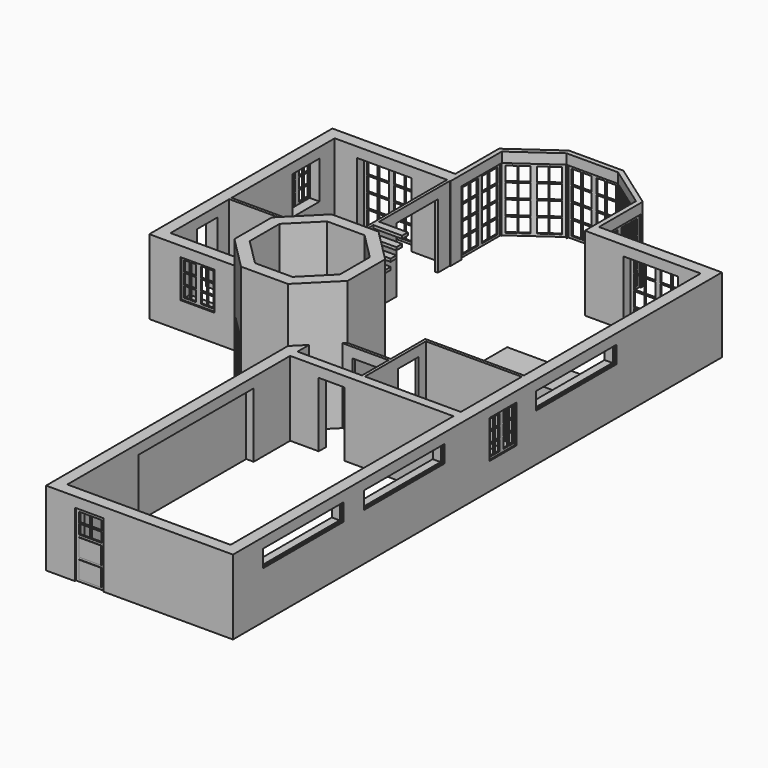
from build123d import *

# Parameters (mm, degrees)
F0_W      = 35.56
F0_H      = 39.9520411314
F1_DEPTH  = 66.04
F2_DEPTH  = 22.86
F3_DEPTH  = 114.3
F4_W      = 23.876
F4_H      = 56.388
F4_W_2    = 19.812
F4_H_2    = 15.24
F4_W_3    = 9.5885
F4_H_3    = 8.5725
F5_DEPTH  = 10.16
F6_START  = -1.27
F6_DEPTH  = 1.27
F7_START  = -0.889
F7_DEPTH  = 1.651
F8_W      = 127
F8_H      = 57.15
F8_W_2    = 16.2983333333
F8_H_2    = 7.9375
F9_DEPTH  = 10.414
F10_START = -1.27
F10_DEPTH = 2.54
F11_START = -1.143
F11_DEPTH = 2.667
F12_W     = 29.972
F12_H     = 33.528
F12_W_2   = 13.8447387577
F12_H_2   = 32.004
F12_W_3   = 13.8412612423
F12_W_4   = 5.08
F12_H_3   = 9.398
F12_W_5   = 5.0673
F12_W_6   = 5.0563387577
F12_W_7   = 5.0436387577
F12_W_8   = 0.762
F12_W_9   = 0.635
F12_H_4   = 0.635
F13_DEPTH = 10.414
F14_START = -1.27
F14_DEPTH = 1.27
F15_W     = 29.972
F15_H     = 33.528
F15_W_2   = 13.8447387577
F15_H_2   = 32.004
F15_W_3   = 13.8412612423
F15_W_4   = 5.08
F15_H_3   = 9.398
F15_W_5   = 5.0673
F15_W_6   = 5.0563387577
F15_W_7   = 5.0436387577
F15_W_8   = 0.762
F15_W_9   = 0.635
F15_H_4   = 0.635
F16_DEPTH = 10.414
F17_START = -1.27
F17_DEPTH = 1.27
F15_W_10  = 22.86
F15_H_5   = 57.15
F18_DEPTH = 10.414
F19_W     = 0.254
F19_H     = 56.388
F19_W_2   = 9.271
F19_H_2   = 12.60475
F20_DEPTH = 10.414
F19_W_3   = 23.241
F21_DEPTH = 10.414
F22_START = -1.27
F22_DEPTH = 1.27
F23_W     = 21.463
F23_H     = 56.388
F23_W_2   = 8.8565006485
F23_H_2   = 12.60475
F23_W_3   = 8.382
F23_W_4   = 7.9074993515
F23_W_5   = 0.254
F24_DEPTH = 4.2164
F25_START = -1.27
F25_DEPTH = 1.27
F26_W     = 21.463
F26_H     = 56.388
F26_W_2   = 8.8565006485
F26_H_2   = 12.60475
F26_W_3   = 8.382
F26_W_4   = 7.9074993515
F26_W_5   = 0.254
F27_DEPTH = 4.2164
F28_START = -1.27
F28_DEPTH = 1.27
F29_W     = 21.463
F29_H     = 56.388
F29_W_2   = 0.254
F29_W_3   = 8.8565006485
F29_H_2   = 12.60475
F29_W_4   = 7.9074993515
F29_W_5   = 8.382
F30_DEPTH = 4.2164
F31_START = -1.27
F31_DEPTH = 1.27
F32_W     = 21.463
F32_H     = 56.388
F32_W_2   = 0.254
F32_W_3   = 8.8565006485
F32_H_2   = 12.60475
F32_W_4   = 7.9074993515
F32_W_5   = 8.382
F33_DEPTH = 4.2164
F34_START = -1.27
F34_DEPTH = 1.27
F35_W     = 21.463
F35_H     = 56.388
F35_W_2   = 0.254
F35_W_3   = 8.8565006485
F35_H_2   = 12.60475
F35_W_4   = 7.9074993515
F35_W_5   = 8.382
F36_DEPTH = 4.2164
F37_START = -1.27
F37_DEPTH = 1.27
F38_W     = 88.9
F38_H     = 15.24
F38_W_2   = 87.376
F38_H_2   = 13.716
F38_W_3   = 29.972
F38_H_3   = 33.528
F38_W_4   = 13.8447387577
F38_H_4   = 32.004
F38_W_5   = 0.762
F38_W_6   = 13.8412612423
F38_W_7   = 5.0563387577
F38_H_5   = 9.398
F38_W_8   = 0.635
F38_W_9   = 5.0673
F38_H_6   = 0.635
F38_W_10  = 5.08
F38_W_11  = 5.0436387577
F39_DEPTH = 10.414
F40_START = -1.27
F40_DEPTH = 1.27
F41_W     = 23.876
F41_H     = 56.388
F41_W_2   = 19.812
F41_H_2   = 15.24
F41_W_3   = 9.5885
F41_H_3   = 8.5725
F42_DEPTH = 10.414
F43_START = -1.27
F43_DEPTH = 3.048
F44_START = -1.27
F44_DEPTH = 1.27
F45_START = -0.889
F45_DEPTH = 1.651
F46_W     = 22.86
F46_H     = 57.15
F47_DEPTH = 50.8
F48_W     = 22.86
F48_H     = 57.15
F49_DEPTH = 2.54
F51_W     = 30.48
F51_H     = 57.15
F52_DEPTH = 10.16
F53_W     = 22.86
F53_H     = 57.15
F54_DEPTH = 2.54
F55_W     = 22.5007897552
F55_H     = 57.15
F56_DEPTH = 10.16
F57_W     = 6.35
F57_H     = 2.54
F58_DEPTH = 25.4
F59_W     = 45.72
F59_H     = 57.15
F60_DEPTH = 2.54


# Not quite as in the source:
# - a feature names something its author has since deleted; it is built from what else it names


with BuildPart() as f1:
    # F0 (on Top) → F1 (new body)
    with BuildSketch(Plane.XY):
        Polygon((0, -540.004), (0, 0), (-108.585, 0), (-108.585, 48.2684106882), (-147.9507946559, 76.2), (-196.2192053441, 76.2), (-235.585, 48.2684106882), (-235.585, 0), (-344.17, 0), (-344.17, -202.184), (-235.8370757085, -202.184), (-225.4230757085, -191.77), (-333.756, -191.77), (-333.756, -126.9259588686), (-333.756, -124.3859588686), (-333.756, -10.414), (-234.4768195874, -10.414), (-231.9368195874, -10.414), (-231.3686, -10.414), (-231.3686, 46.0901700506), (-194.875315105, 71.9836), (-149.294684895, 71.9836), (-112.8014, 46.0901700506), (-112.8014, -10.414), (-10.414, -10.414), (-10.414, -115.0290641975), (-10.414, -205.5208195874), (-10.414, -208.0608195874), (-10.414, -275.336), (-10.414, -283.464), (-10.414, -529.59), (-154.686, -529.59), (-154.686, -283.464), (-154.686, -275.336), (-154.686, -262.5070757085), (-165.1, -272.9210757085), (-165.1, -540.004), align=None)
        Polygon((-234.4768195874, -10.414), (-234.4768195874, -124.3859588686), (-231.9368195874, -124.3859588686), (-231.9368195874, -103.886), (-231.9368195874, -10.414), align=None)
        Polygon((-272.5768195874, -169.418), (-215.9541536726, -169.418), (-206.5368195874, -169.418), (-206.5368195874, -166.878), (-231.9368195874, -166.878), (-231.9368195874, -124.3859588686), (-234.4768195874, -124.3859588686), (-333.756, -124.3859588686), (-333.756, -126.9259588686), (-272.5768195874, -126.9259588686), align=None)
        with Locations((-252.2568195874, -146.9019794343)):
            Rectangle(F0_W, F0_H, mode=Mode.SUBTRACT)
        Polygon((-215.9541536726, -169.418), (-209.5126146906, -175.8595389821), (-206.5368195874, -172.8837438789), (-206.5368195874, -169.418), align=None)
        Polygon((-97.6997438789, -243.6208195874), (-97.6997438789, -246.1608195874), (-97.6997438789, -275.336), (-95.1597438789, -275.336), (-95.1597438789, -208.0608195874), (-10.414, -208.0608195874), (-10.414, -205.5208195874), (-97.6997438789, -205.5208195874), align=None)
        Polygon((-135.7997438789, -243.6208195874), (-138.3397438789, -246.1608195874), (-97.6997438789, -246.1608195874), (-97.6997438789, -243.6208195874), align=None)
        Polygon((-97.6997438789, -275.336), (-154.686, -275.336), (-154.686, -283.464), (-10.414, -283.464), (-10.414, -275.336), (-95.1597438789, -275.336), align=None)
    extrude(amount=F1_DEPTH)

    # F0 (on Top) → F2 (join)
    with BuildSketch(Plane.XY):
        Polygon((-97.6997438789, -190.2808195874), (-97.6997438789, -205.5208195874), (-10.414, -205.5208195874), (-10.414, -115.0290641975), (-97.6997438789, -115.0290641975), (-97.6997438789, -145.5090641975), (-25.654, -145.5090641975), (-25.654, -190.2808195874), align=None)
    extrude(amount=F2_DEPTH)

    # F0 (on Top) → F3 (join)
    with BuildSketch(Plane.XY):
        Polygon((-206.5368195874, -272.9210757085), (-165.1, -272.9210757085), (-154.686, -262.5070757085), (-138.3397438789, -246.1608195874), (-135.7997438789, -243.6208195874), (-135.7997438789, -202.184), (-165.1, -172.8837438789), (-206.5368195874, -172.8837438789), (-209.5126146906, -175.8595389821), (-225.4230757085, -191.77), (-235.8370757085, -202.184), (-235.8370757085, -243.6208195874), align=None)
        Polygon((-202.3284097937, -262.7610757085), (-225.6770757085, -239.4124097937), (-225.6770757085, -206.3924097937), (-202.3284097937, -183.0437438789), (-169.3084097937, -183.0437438789), (-145.9597438789, -206.3924097937), (-145.9597438789, -239.4124097937), (-169.3084097937, -262.7610757085), align=None, mode=Mode.SUBTRACT)
    extrude(amount=F3_DEPTH)

    # F4 (on face) → F5 (cut)
    with BuildSketch(Plane(origin=(-239.728947648, -239.728947648, 0), x_dir=(0.7071067812, -0.7071067812, 0), z_dir=(-0.7071067812, -0.7071067812, 0))):
        Polygon((13.5397576672, 57.15), (13.5397576672, 0), (14.3017576672, 0), (14.3017576672, 56.388), (38.1777576672, 56.388), (38.1777576672, 0), (38.9397576672, 0), (38.9397576672, 57.15), align=None)
        with Locations((26.2397576672, 28.194)):
            Rectangle(F4_W, F4_H)
        with Locations((26.2397576672, 26.924)):
            Rectangle(F4_W_2, F4_H_2, mode=Mode.SUBTRACT)
        with Locations((26.2397576672, 9.652)):
            Rectangle(F4_W_2, F4_H_2, mode=Mode.SUBTRACT)
        with Locations((21.1280076672, 40.86225)):
            Rectangle(F4_W_3, F4_H_3, mode=Mode.SUBTRACT)
        with Locations((21.1280076672, 50.06975)):
            Rectangle(F4_W_3, F4_H_3, mode=Mode.SUBTRACT)
        with Locations((31.3515076672, 40.86225)):
            Rectangle(F4_W_3, F4_H_3, mode=Mode.SUBTRACT)
        with Locations((31.3515076672, 50.06975)):
            Rectangle(F4_W_3, F4_H_3, mode=Mode.SUBTRACT)
        with Locations((21.1280076672, 50.06975)):
            Rectangle(F4_W_3, F4_H_3)
        with Locations((31.3515076672, 50.06975)):
            Rectangle(F4_W_3, F4_H_3)
        with Locations((31.3515076672, 40.86225)):
            Rectangle(F4_W_3, F4_H_3)
        with Locations((21.1280076672, 40.86225)):
            Rectangle(F4_W_3, F4_H_3)
        with Locations((26.2397576672, 26.924)):
            Rectangle(F4_W_2, F4_H_2)
        with Locations((26.2397576672, 9.652)):
            Rectangle(F4_W_2, F4_H_2)
    extrude(amount=-F5_DEPTH, mode=Mode.SUBTRACT)

    # F4 (on face) → F6 (join)
    with BuildSketch(Plane(origin=(-239.728947648, -239.728947648, 0), x_dir=(0.7071067812, -0.7071067812, 0), z_dir=(-0.7071067812, -0.7071067812, 0)).offset(F6_START)):
        Polygon((13.5397576672, 57.15), (13.5397576672, 0), (14.3017576672, 0), (14.3017576672, 56.388), (38.1777576672, 56.388), (38.1777576672, 0), (38.9397576672, 0), (38.9397576672, 57.15), align=None)
        with Locations((26.2397576672, 28.194)):
            Rectangle(F4_W, F4_H)
        with Locations((26.2397576672, 26.924)):
            Rectangle(F4_W_2, F4_H_2, mode=Mode.SUBTRACT)
        with Locations((26.2397576672, 9.652)):
            Rectangle(F4_W_2, F4_H_2, mode=Mode.SUBTRACT)
        with Locations((21.1280076672, 40.86225)):
            Rectangle(F4_W_3, F4_H_3, mode=Mode.SUBTRACT)
        with Locations((21.1280076672, 50.06975)):
            Rectangle(F4_W_3, F4_H_3, mode=Mode.SUBTRACT)
        with Locations((31.3515076672, 40.86225)):
            Rectangle(F4_W_3, F4_H_3, mode=Mode.SUBTRACT)
        with Locations((31.3515076672, 50.06975)):
            Rectangle(F4_W_3, F4_H_3, mode=Mode.SUBTRACT)
    extrude(amount=-F6_DEPTH)

    # F4 (on face) → F7 (join)
    with BuildSketch(Plane(origin=(-239.728947648, -239.728947648, 0), x_dir=(0.7071067812, -0.7071067812, 0), z_dir=(-0.7071067812, -0.7071067812, 0)).offset(F7_START)):
        with Locations((26.2397576672, 26.924)):
            Rectangle(F4_W_2, F4_H_2)
        with Locations((26.2397576672, 9.652)):
            Rectangle(F4_W_2, F4_H_2)
    extrude(amount=-F7_DEPTH)

    # F8 (on face) → F9 (cut)
    with BuildSketch(Plane(origin=(-165.1, 0, 0), x_dir=(0, -1, 0), z_dir=(-1, 0, 0))):
        with Locations((387.2210757085, 28.575)):
            Rectangle(F8_W, F8_H)
        with Locations((336.9502423752, 11.58875)):
            Rectangle(F8_W_2, F8_H_2, mode=Mode.SUBTRACT)
        with Locations((357.0585757085, 11.58875)):
            Rectangle(F8_W_2, F8_H_2, mode=Mode.SUBTRACT)
        with Locations((377.1669090418, 11.58875)):
            Rectangle(F8_W_2, F8_H_2, mode=Mode.SUBTRACT)
        with Locations((397.2752423752, 11.58875)):
            Rectangle(F8_W_2, F8_H_2, mode=Mode.SUBTRACT)
        with Locations((336.9502423752, 23.33625)):
            Rectangle(F8_W_2, F8_H_2, mode=Mode.SUBTRACT)
        with Locations((357.0585757085, 23.33625)):
            Rectangle(F8_W_2, F8_H_2, mode=Mode.SUBTRACT)
        with Locations((377.1669090418, 23.33625)):
            Rectangle(F8_W_2, F8_H_2, mode=Mode.SUBTRACT)
        with Locations((397.2752423752, 23.33625)):
            Rectangle(F8_W_2, F8_H_2, mode=Mode.SUBTRACT)
        with Locations((417.3835757085, 11.58875)):
            Rectangle(F8_W_2, F8_H_2, mode=Mode.SUBTRACT)
        with Locations((437.4919090418, 11.58875)):
            Rectangle(F8_W_2, F8_H_2, mode=Mode.SUBTRACT)
        with Locations((417.3835757085, 23.33625)):
            Rectangle(F8_W_2, F8_H_2, mode=Mode.SUBTRACT)
        with Locations((437.4919090418, 23.33625)):
            Rectangle(F8_W_2, F8_H_2, mode=Mode.SUBTRACT)
        with Locations((336.9502423752, 36.35375)):
            Rectangle(F8_W_2, F8_H_2, mode=Mode.SUBTRACT)
        with Locations((336.9502423752, 48.10125)):
            Rectangle(F8_W_2, F8_H_2, mode=Mode.SUBTRACT)
        with Locations((357.0585757085, 36.35375)):
            Rectangle(F8_W_2, F8_H_2, mode=Mode.SUBTRACT)
        with Locations((377.1669090418, 36.35375)):
            Rectangle(F8_W_2, F8_H_2, mode=Mode.SUBTRACT)
        with Locations((397.2752423752, 36.35375)):
            Rectangle(F8_W_2, F8_H_2, mode=Mode.SUBTRACT)
        with Locations((357.0585757085, 48.10125)):
            Rectangle(F8_W_2, F8_H_2, mode=Mode.SUBTRACT)
        with Locations((377.1669090418, 48.10125)):
            Rectangle(F8_W_2, F8_H_2, mode=Mode.SUBTRACT)
        with Locations((397.2752423752, 48.10125)):
            Rectangle(F8_W_2, F8_H_2, mode=Mode.SUBTRACT)
        with Locations((417.3835757085, 36.35375)):
            Rectangle(F8_W_2, F8_H_2, mode=Mode.SUBTRACT)
        with Locations((437.4919090418, 36.35375)):
            Rectangle(F8_W_2, F8_H_2, mode=Mode.SUBTRACT)
        with Locations((417.3835757085, 48.10125)):
            Rectangle(F8_W_2, F8_H_2, mode=Mode.SUBTRACT)
        with Locations((437.4919090418, 48.10125)):
            Rectangle(F8_W_2, F8_H_2, mode=Mode.SUBTRACT)
        with Locations((336.9502423752, 48.10125)):
            Rectangle(F8_W_2, F8_H_2)
        with Locations((357.0585757085, 48.10125)):
            Rectangle(F8_W_2, F8_H_2)
        with Locations((377.1669090418, 48.10125)):
            Rectangle(F8_W_2, F8_H_2)
        with Locations((397.2752423752, 48.10125)):
            Rectangle(F8_W_2, F8_H_2)
        with Locations((417.3835757085, 48.10125)):
            Rectangle(F8_W_2, F8_H_2)
        with Locations((437.4919090418, 48.10125)):
            Rectangle(F8_W_2, F8_H_2)
        with Locations((336.9502423752, 36.35375)):
            Rectangle(F8_W_2, F8_H_2)
        with Locations((357.0585757085, 36.35375)):
            Rectangle(F8_W_2, F8_H_2)
        with Locations((377.1669090418, 36.35375)):
            Rectangle(F8_W_2, F8_H_2)
        with Locations((397.2752423752, 36.35375)):
            Rectangle(F8_W_2, F8_H_2)
        with Locations((417.3835757085, 36.35375)):
            Rectangle(F8_W_2, F8_H_2)
        with Locations((437.4919090418, 36.35375)):
            Rectangle(F8_W_2, F8_H_2)
        with Locations((336.9502423752, 23.33625)):
            Rectangle(F8_W_2, F8_H_2)
        with Locations((357.0585757085, 23.33625)):
            Rectangle(F8_W_2, F8_H_2)
        with Locations((377.1669090418, 23.33625)):
            Rectangle(F8_W_2, F8_H_2)
        with Locations((397.2752423752, 23.33625)):
            Rectangle(F8_W_2, F8_H_2)
        with Locations((417.3835757085, 23.33625)):
            Rectangle(F8_W_2, F8_H_2)
        with Locations((437.4919090418, 23.33625)):
            Rectangle(F8_W_2, F8_H_2)
        with Locations((336.9502423752, 11.58875)):
            Rectangle(F8_W_2, F8_H_2)
        with Locations((357.0585757085, 11.58875)):
            Rectangle(F8_W_2, F8_H_2)
        with Locations((377.1669090418, 11.58875)):
            Rectangle(F8_W_2, F8_H_2)
        with Locations((397.2752423752, 11.58875)):
            Rectangle(F8_W_2, F8_H_2)
        with Locations((417.3835757085, 11.58875)):
            Rectangle(F8_W_2, F8_H_2)
        with Locations((437.4919090418, 11.58875)):
            Rectangle(F8_W_2, F8_H_2)
    extrude(amount=-F9_DEPTH, mode=Mode.SUBTRACT)

    # F8 (on face) → F10 (join)
    with BuildSketch(Plane(origin=(-165.1, 0, 0), x_dir=(0, -1, 0), z_dir=(-1, 0, 0)).offset(F10_START)):
        with Locations((387.2210757085, 28.575)):
            Rectangle(F8_W, F8_H)
        with Locations((336.9502423752, 11.58875)):
            Rectangle(F8_W_2, F8_H_2, mode=Mode.SUBTRACT)
        with Locations((357.0585757085, 11.58875)):
            Rectangle(F8_W_2, F8_H_2, mode=Mode.SUBTRACT)
        with Locations((377.1669090418, 11.58875)):
            Rectangle(F8_W_2, F8_H_2, mode=Mode.SUBTRACT)
        with Locations((397.2752423752, 11.58875)):
            Rectangle(F8_W_2, F8_H_2, mode=Mode.SUBTRACT)
        with Locations((336.9502423752, 23.33625)):
            Rectangle(F8_W_2, F8_H_2, mode=Mode.SUBTRACT)
        with Locations((357.0585757085, 23.33625)):
            Rectangle(F8_W_2, F8_H_2, mode=Mode.SUBTRACT)
        with Locations((377.1669090418, 23.33625)):
            Rectangle(F8_W_2, F8_H_2, mode=Mode.SUBTRACT)
        with Locations((397.2752423752, 23.33625)):
            Rectangle(F8_W_2, F8_H_2, mode=Mode.SUBTRACT)
        with Locations((417.3835757085, 11.58875)):
            Rectangle(F8_W_2, F8_H_2, mode=Mode.SUBTRACT)
        with Locations((437.4919090418, 11.58875)):
            Rectangle(F8_W_2, F8_H_2, mode=Mode.SUBTRACT)
        with Locations((417.3835757085, 23.33625)):
            Rectangle(F8_W_2, F8_H_2, mode=Mode.SUBTRACT)
        with Locations((437.4919090418, 23.33625)):
            Rectangle(F8_W_2, F8_H_2, mode=Mode.SUBTRACT)
        with Locations((336.9502423752, 36.35375)):
            Rectangle(F8_W_2, F8_H_2, mode=Mode.SUBTRACT)
        with Locations((336.9502423752, 48.10125)):
            Rectangle(F8_W_2, F8_H_2, mode=Mode.SUBTRACT)
        with Locations((357.0585757085, 36.35375)):
            Rectangle(F8_W_2, F8_H_2, mode=Mode.SUBTRACT)
        with Locations((377.1669090418, 36.35375)):
            Rectangle(F8_W_2, F8_H_2, mode=Mode.SUBTRACT)
        with Locations((397.2752423752, 36.35375)):
            Rectangle(F8_W_2, F8_H_2, mode=Mode.SUBTRACT)
        with Locations((357.0585757085, 48.10125)):
            Rectangle(F8_W_2, F8_H_2, mode=Mode.SUBTRACT)
        with Locations((377.1669090418, 48.10125)):
            Rectangle(F8_W_2, F8_H_2, mode=Mode.SUBTRACT)
        with Locations((397.2752423752, 48.10125)):
            Rectangle(F8_W_2, F8_H_2, mode=Mode.SUBTRACT)
        with Locations((417.3835757085, 36.35375)):
            Rectangle(F8_W_2, F8_H_2, mode=Mode.SUBTRACT)
        with Locations((437.4919090418, 36.35375)):
            Rectangle(F8_W_2, F8_H_2, mode=Mode.SUBTRACT)
        with Locations((417.3835757085, 48.10125)):
            Rectangle(F8_W_2, F8_H_2, mode=Mode.SUBTRACT)
        with Locations((437.4919090418, 48.10125)):
            Rectangle(F8_W_2, F8_H_2, mode=Mode.SUBTRACT)
    extrude(amount=-F10_DEPTH)

    # F8 (on face) → F11 (join)
    with BuildSketch(Plane(origin=(-165.1, 0, 0), x_dir=(0, -1, 0), z_dir=(-1, 0, 0)).offset(F11_START)):
        with Locations((336.9502423752, 48.10125)):
            Rectangle(F8_W_2, F8_H_2)
        with Locations((357.0585757085, 48.10125)):
            Rectangle(F8_W_2, F8_H_2)
        with Locations((377.1669090418, 48.10125)):
            Rectangle(F8_W_2, F8_H_2)
        with Locations((397.2752423752, 48.10125)):
            Rectangle(F8_W_2, F8_H_2)
        with Locations((417.3835757085, 48.10125)):
            Rectangle(F8_W_2, F8_H_2)
        with Locations((437.4919090418, 48.10125)):
            Rectangle(F8_W_2, F8_H_2)
        with Locations((336.9502423752, 36.35375)):
            Rectangle(F8_W_2, F8_H_2)
        with Locations((357.0585757085, 36.35375)):
            Rectangle(F8_W_2, F8_H_2)
        with Locations((377.1669090418, 36.35375)):
            Rectangle(F8_W_2, F8_H_2)
        with Locations((397.2752423752, 36.35375)):
            Rectangle(F8_W_2, F8_H_2)
        with Locations((417.3835757085, 36.35375)):
            Rectangle(F8_W_2, F8_H_2)
        with Locations((437.4919090418, 36.35375)):
            Rectangle(F8_W_2, F8_H_2)
        with Locations((336.9502423752, 23.33625)):
            Rectangle(F8_W_2, F8_H_2)
        with Locations((357.0585757085, 23.33625)):
            Rectangle(F8_W_2, F8_H_2)
        with Locations((377.1669090418, 23.33625)):
            Rectangle(F8_W_2, F8_H_2)
        with Locations((397.2752423752, 23.33625)):
            Rectangle(F8_W_2, F8_H_2)
        with Locations((417.3835757085, 23.33625)):
            Rectangle(F8_W_2, F8_H_2)
        with Locations((437.4919090418, 23.33625)):
            Rectangle(F8_W_2, F8_H_2)
        with Locations((336.9502423752, 11.58875)):
            Rectangle(F8_W_2, F8_H_2)
        with Locations((357.0585757085, 11.58875)):
            Rectangle(F8_W_2, F8_H_2)
        with Locations((377.1669090418, 11.58875)):
            Rectangle(F8_W_2, F8_H_2)
        with Locations((397.2752423752, 11.58875)):
            Rectangle(F8_W_2, F8_H_2)
        with Locations((417.3835757085, 11.58875)):
            Rectangle(F8_W_2, F8_H_2)
        with Locations((437.4919090418, 11.58875)):
            Rectangle(F8_W_2, F8_H_2)
    extrude(amount=-F11_DEPTH)

    # F12 (on face) → F13 (cut)
    with BuildSketch(Plane.XZ.offset(202.184)):
        with Locations((-301.6230757085, 40.386)):
            Rectangle(F12_W, F12_H)
        Polygon((-315.8470757085, 24.384), (-315.8470757085, 56.388), (-302.0023369508, 56.388), (-301.2403369508, 56.388), (-287.3990757085, 56.388), (-287.3990757085, 24.384), (-301.2403369508, 24.384), (-302.0023369508, 24.384), align=None, mode=Mode.SUBTRACT)
        with Locations((-308.9247063296, 40.386)):
            Rectangle(F12_W_2, F12_H_2)
        Polygon((-314.5770757085, 45.72), (-314.5770757085, 55.118), (-309.5207369508, 55.118), (-308.8857369508, 55.118), (-303.8184369508, 55.118), (-303.8184369508, 45.72), (-303.8184369508, 45.085), (-303.8184369508, 35.687), (-303.8184369508, 35.052), (-303.8184369508, 25.654), (-308.8857369508, 25.654), (-309.5207369508, 25.654), (-314.5770757085, 25.654), (-314.5770757085, 35.052), (-314.5770757085, 35.687), (-314.5770757085, 45.085), align=None, mode=Mode.SUBTRACT)
        with Locations((-294.3197063296, 40.386)):
            Rectangle(F12_W_3, F12_H_2)
        Polygon((-299.4277144662, 45.72), (-299.4277144662, 55.118), (-294.3477144662, 55.118), (-293.7127144662, 55.118), (-288.6690757085, 55.118), (-288.6690757085, 45.72), (-288.6690757085, 45.085), (-288.6690757085, 35.687), (-288.6690757085, 35.052), (-288.6690757085, 25.654), (-293.7127144662, 25.654), (-294.3477144662, 25.654), (-299.4277144662, 25.654), (-299.4277144662, 35.052), (-299.4277144662, 35.687), (-299.4277144662, 45.085), align=None, mode=Mode.SUBTRACT)
        with Locations((-296.8877144662, 30.353)):
            Rectangle(F12_W_4, F12_H_3)
        with Locations((-296.8877144662, 40.386)):
            Rectangle(F12_W_4, F12_H_3)
        with Locations((-296.8877144662, 50.419)):
            Rectangle(F12_W_4, F12_H_3)
        with Locations((-306.3520869508, 50.419)):
            Rectangle(F12_W_5, F12_H_3)
        with Locations((-306.3520869508, 40.386)):
            Rectangle(F12_W_5, F12_H_3)
        with Locations((-306.3520869508, 30.353)):
            Rectangle(F12_W_5, F12_H_3)
        with Locations((-312.0489063296, 50.419)):
            Rectangle(F12_W_6, F12_H_3)
        with Locations((-312.0489063296, 40.386)):
            Rectangle(F12_W_6, F12_H_3)
        with Locations((-312.0489063296, 30.353)):
            Rectangle(F12_W_6, F12_H_3)
        with Locations((-291.1908950873, 30.353)):
            Rectangle(F12_W_7, F12_H_3)
        with Locations((-291.1908950873, 40.386)):
            Rectangle(F12_W_7, F12_H_3)
        with Locations((-291.1908950873, 50.419)):
            Rectangle(F12_W_7, F12_H_3)
        with Locations((-301.6213369508, 40.386)):
            Rectangle(F12_W_8, F12_H_2)
        with Locations((-294.0302144662, 50.419)):
            Rectangle(F12_W_9, F12_H_3)
        with Locations((-294.0302144662, 40.386)):
            Rectangle(F12_W_9, F12_H_3)
        with Locations((-309.2032369508, 50.419)):
            Rectangle(F12_W_9, F12_H_3)
        with Locations((-309.2032369508, 40.386)):
            Rectangle(F12_W_9, F12_H_3)
        with Locations((-294.0302144662, 30.353)):
            Rectangle(F12_W_9, F12_H_3)
        with Locations((-309.2032369508, 30.353)):
            Rectangle(F12_W_9, F12_H_3)
        with Locations((-296.8877144662, 45.4025)):
            Rectangle(F12_W_4, F12_H_4)
        with Locations((-296.8877144662, 35.3695)):
            Rectangle(F12_W_4, F12_H_4)
        with Locations((-306.3520869508, 45.4025)):
            Rectangle(F12_W_5, F12_H_4)
        with Locations((-306.3520869508, 35.3695)):
            Rectangle(F12_W_5, F12_H_4)
        with Locations((-312.0489063296, 45.4025)):
            Rectangle(F12_W_6, F12_H_4)
        with Locations((-312.0489063296, 35.3695)):
            Rectangle(F12_W_6, F12_H_4)
        with Locations((-291.1908950873, 45.4025)):
            Rectangle(F12_W_7, F12_H_4)
        with Locations((-291.1908950873, 35.3695)):
            Rectangle(F12_W_7, F12_H_4)
        with Locations((-294.0302144662, 45.4025)):
            Rectangle(F12_W_9, F12_H_4)
        with Locations((-309.2032369508, 45.4025)):
            Rectangle(F12_W_9, F12_H_4)
        with Locations((-294.0302144662, 35.3695)):
            Rectangle(F12_W_9, F12_H_4)
        with Locations((-309.2032369508, 35.3695)):
            Rectangle(F12_W_9, F12_H_4)
    extrude(amount=-F13_DEPTH, mode=Mode.SUBTRACT)

    # F12 (on face) → F14 (join)
    with BuildSketch(Plane.XZ.offset(202.184).offset(F14_START)):
        with Locations((-301.6230757085, 40.386)):
            Rectangle(F12_W, F12_H)
        Polygon((-315.8470757085, 24.384), (-315.8470757085, 56.388), (-302.0023369508, 56.388), (-301.2403369508, 56.388), (-287.3990757085, 56.388), (-287.3990757085, 24.384), (-301.2403369508, 24.384), (-302.0023369508, 24.384), align=None, mode=Mode.SUBTRACT)
        with Locations((-308.9247063296, 40.386)):
            Rectangle(F12_W_2, F12_H_2)
        Polygon((-314.5770757085, 45.72), (-314.5770757085, 55.118), (-309.5207369508, 55.118), (-308.8857369508, 55.118), (-303.8184369508, 55.118), (-303.8184369508, 45.72), (-303.8184369508, 45.085), (-303.8184369508, 35.687), (-303.8184369508, 35.052), (-303.8184369508, 25.654), (-308.8857369508, 25.654), (-309.5207369508, 25.654), (-314.5770757085, 25.654), (-314.5770757085, 35.052), (-314.5770757085, 35.687), (-314.5770757085, 45.085), align=None, mode=Mode.SUBTRACT)
        with Locations((-294.3197063296, 40.386)):
            Rectangle(F12_W_3, F12_H_2)
        Polygon((-299.4277144662, 45.72), (-299.4277144662, 55.118), (-294.3477144662, 55.118), (-293.7127144662, 55.118), (-288.6690757085, 55.118), (-288.6690757085, 45.72), (-288.6690757085, 45.085), (-288.6690757085, 35.687), (-288.6690757085, 35.052), (-288.6690757085, 25.654), (-293.7127144662, 25.654), (-294.3477144662, 25.654), (-299.4277144662, 25.654), (-299.4277144662, 35.052), (-299.4277144662, 35.687), (-299.4277144662, 45.085), align=None, mode=Mode.SUBTRACT)
        with Locations((-301.6213369508, 40.386)):
            Rectangle(F12_W_8, F12_H_2)
        with Locations((-309.2032369508, 50.419)):
            Rectangle(F12_W_9, F12_H_3)
        with Locations((-309.2032369508, 40.386)):
            Rectangle(F12_W_9, F12_H_3)
        with Locations((-294.0302144662, 50.419)):
            Rectangle(F12_W_9, F12_H_3)
        with Locations((-294.0302144662, 40.386)):
            Rectangle(F12_W_9, F12_H_3)
        with Locations((-309.2032369508, 30.353)):
            Rectangle(F12_W_9, F12_H_3)
        with Locations((-294.0302144662, 30.353)):
            Rectangle(F12_W_9, F12_H_3)
        with Locations((-296.8877144662, 45.4025)):
            Rectangle(F12_W_4, F12_H_4)
        with Locations((-296.8877144662, 35.3695)):
            Rectangle(F12_W_4, F12_H_4)
        with Locations((-306.3520869508, 45.4025)):
            Rectangle(F12_W_5, F12_H_4)
        with Locations((-306.3520869508, 35.3695)):
            Rectangle(F12_W_5, F12_H_4)
        with Locations((-312.0489063296, 45.4025)):
            Rectangle(F12_W_6, F12_H_4)
        with Locations((-312.0489063296, 35.3695)):
            Rectangle(F12_W_6, F12_H_4)
        with Locations((-291.1908950873, 45.4025)):
            Rectangle(F12_W_7, F12_H_4)
        with Locations((-291.1908950873, 35.3695)):
            Rectangle(F12_W_7, F12_H_4)
        with Locations((-309.2032369508, 45.4025)):
            Rectangle(F12_W_9, F12_H_4)
        with Locations((-294.0302144662, 45.4025)):
            Rectangle(F12_W_9, F12_H_4)
        with Locations((-309.2032369508, 35.3695)):
            Rectangle(F12_W_9, F12_H_4)
        with Locations((-294.0302144662, 35.3695)):
            Rectangle(F12_W_9, F12_H_4)
    extrude(amount=-F14_DEPTH)

    # F15 (on face) → F16 (cut)
    with BuildSketch(Plane(origin=(-344.17, 0, 0), x_dir=(0, -1, 0), z_dir=(-1, 0, 0))):
        with Locations((42.164, 40.386)):
            Rectangle(F15_W, F15_H)
        Polygon((27.94, 24.384), (27.94, 56.388), (41.7847387577, 56.388), (42.5467387577, 56.388), (56.388, 56.388), (56.388, 24.384), (42.5467387577, 24.384), (41.7847387577, 24.384), align=None, mode=Mode.SUBTRACT)
        with Locations((34.8623693789, 40.386)):
            Rectangle(F15_W_2, F15_H_2)
        Polygon((29.21, 45.72), (29.21, 55.118), (34.2663387577, 55.118), (34.9013387577, 55.118), (39.9686387577, 55.118), (39.9686387577, 45.72), (39.9686387577, 45.085), (39.9686387577, 35.687), (39.9686387577, 35.052), (39.9686387577, 25.654), (34.9013387577, 25.654), (34.2663387577, 25.654), (29.21, 25.654), (29.21, 35.052), (29.21, 35.687), (29.21, 45.085), align=None, mode=Mode.SUBTRACT)
        with Locations((49.4673693789, 40.386)):
            Rectangle(F15_W_3, F15_H_2)
        Polygon((44.3593612423, 45.72), (44.3593612423, 55.118), (49.4393612423, 55.118), (50.0743612423, 55.118), (55.118, 55.118), (55.118, 45.72), (55.118, 45.085), (55.118, 35.687), (55.118, 35.052), (55.118, 25.654), (50.0743612423, 25.654), (49.4393612423, 25.654), (44.3593612423, 25.654), (44.3593612423, 35.052), (44.3593612423, 35.687), (44.3593612423, 45.085), align=None, mode=Mode.SUBTRACT)
        with Locations((46.8993612423, 50.419)):
            Rectangle(F15_W_4, F15_H_3)
        with Locations((46.8993612423, 40.386)):
            Rectangle(F15_W_4, F15_H_3)
        with Locations((46.8993612423, 30.353)):
            Rectangle(F15_W_4, F15_H_3)
        with Locations((37.4349887577, 50.419)):
            Rectangle(F15_W_5, F15_H_3)
        with Locations((37.4349887577, 40.386)):
            Rectangle(F15_W_5, F15_H_3)
        with Locations((37.4349887577, 30.353)):
            Rectangle(F15_W_5, F15_H_3)
        with Locations((31.7381693789, 50.419)):
            Rectangle(F15_W_6, F15_H_3)
        with Locations((31.7381693789, 40.386)):
            Rectangle(F15_W_6, F15_H_3)
        with Locations((31.7381693789, 30.353)):
            Rectangle(F15_W_6, F15_H_3)
        with Locations((52.5961806211, 50.419)):
            Rectangle(F15_W_7, F15_H_3)
        with Locations((52.5961806211, 40.386)):
            Rectangle(F15_W_7, F15_H_3)
        with Locations((52.5961806211, 30.353)):
            Rectangle(F15_W_7, F15_H_3)
        with Locations((42.1657387577, 40.386)):
            Rectangle(F15_W_8, F15_H_2)
        with Locations((34.5838387577, 50.419)):
            Rectangle(F15_W_9, F15_H_3)
        with Locations((34.5838387577, 40.386)):
            Rectangle(F15_W_9, F15_H_3)
        with Locations((34.5838387577, 30.353)):
            Rectangle(F15_W_9, F15_H_3)
        with Locations((49.7568612423, 50.419)):
            Rectangle(F15_W_9, F15_H_3)
        with Locations((49.7568612423, 40.386)):
            Rectangle(F15_W_9, F15_H_3)
        with Locations((49.7568612423, 30.353)):
            Rectangle(F15_W_9, F15_H_3)
        with Locations((46.8993612423, 45.4025)):
            Rectangle(F15_W_4, F15_H_4)
        with Locations((46.8993612423, 35.3695)):
            Rectangle(F15_W_4, F15_H_4)
        with Locations((37.4349887577, 45.4025)):
            Rectangle(F15_W_5, F15_H_4)
        with Locations((37.4349887577, 35.3695)):
            Rectangle(F15_W_5, F15_H_4)
        with Locations((31.7381693789, 45.4025)):
            Rectangle(F15_W_6, F15_H_4)
        with Locations((31.7381693789, 35.3695)):
            Rectangle(F15_W_6, F15_H_4)
        with Locations((52.5961806211, 45.4025)):
            Rectangle(F15_W_7, F15_H_4)
        with Locations((52.5961806211, 35.3695)):
            Rectangle(F15_W_7, F15_H_4)
        with Locations((34.5838387577, 45.4025)):
            Rectangle(F15_W_9, F15_H_4)
        with Locations((34.5838387577, 35.3695)):
            Rectangle(F15_W_9, F15_H_4)
        with Locations((49.7568612423, 45.4025)):
            Rectangle(F15_W_9, F15_H_4)
        with Locations((49.7568612423, 35.3695)):
            Rectangle(F15_W_9, F15_H_4)
    extrude(amount=-F16_DEPTH, mode=Mode.SUBTRACT)

    # F15 (on face) → F17 (join)
    with BuildSketch(Plane(origin=(-344.17, 0, 0), x_dir=(0, -1, 0), z_dir=(-1, 0, 0)).offset(F17_START)):
        with Locations((42.164, 40.386)):
            Rectangle(F15_W, F15_H)
        Polygon((27.94, 24.384), (27.94, 56.388), (41.7847387577, 56.388), (42.5467387577, 56.388), (56.388, 56.388), (56.388, 24.384), (42.5467387577, 24.384), (41.7847387577, 24.384), align=None, mode=Mode.SUBTRACT)
        with Locations((34.8623693789, 40.386)):
            Rectangle(F15_W_2, F15_H_2)
        Polygon((29.21, 45.72), (29.21, 55.118), (34.2663387577, 55.118), (34.9013387577, 55.118), (39.9686387577, 55.118), (39.9686387577, 45.72), (39.9686387577, 45.085), (39.9686387577, 35.687), (39.9686387577, 35.052), (39.9686387577, 25.654), (34.9013387577, 25.654), (34.2663387577, 25.654), (29.21, 25.654), (29.21, 35.052), (29.21, 35.687), (29.21, 45.085), align=None, mode=Mode.SUBTRACT)
        with Locations((42.1657387577, 40.386)):
            Rectangle(F15_W_8, F15_H_2)
        with Locations((49.4673693789, 40.386)):
            Rectangle(F15_W_3, F15_H_2)
        Polygon((44.3593612423, 45.72), (44.3593612423, 55.118), (49.4393612423, 55.118), (50.0743612423, 55.118), (55.118, 55.118), (55.118, 45.72), (55.118, 45.085), (55.118, 35.687), (55.118, 35.052), (55.118, 25.654), (50.0743612423, 25.654), (49.4393612423, 25.654), (44.3593612423, 25.654), (44.3593612423, 35.052), (44.3593612423, 35.687), (44.3593612423, 45.085), align=None, mode=Mode.SUBTRACT)
        with Locations((49.7568612423, 50.419)):
            Rectangle(F15_W_9, F15_H_3)
        with Locations((49.7568612423, 45.4025)):
            Rectangle(F15_W_9, F15_H_4)
        with Locations((52.5961806211, 45.4025)):
            Rectangle(F15_W_7, F15_H_4)
        with Locations((46.8993612423, 45.4025)):
            Rectangle(F15_W_4, F15_H_4)
        with Locations((49.7568612423, 40.386)):
            Rectangle(F15_W_9, F15_H_3)
        with Locations((52.5961806211, 35.3695)):
            Rectangle(F15_W_7, F15_H_4)
        with Locations((49.7568612423, 30.353)):
            Rectangle(F15_W_9, F15_H_3)
        with Locations((49.7568612423, 35.3695)):
            Rectangle(F15_W_9, F15_H_4)
        with Locations((46.8993612423, 35.3695)):
            Rectangle(F15_W_4, F15_H_4)
        with Locations((37.4349887577, 35.3695)):
            Rectangle(F15_W_5, F15_H_4)
        with Locations((34.5838387577, 35.3695)):
            Rectangle(F15_W_9, F15_H_4)
        with Locations((31.7381693789, 35.3695)):
            Rectangle(F15_W_6, F15_H_4)
        with Locations((34.5838387577, 40.386)):
            Rectangle(F15_W_9, F15_H_3)
        with Locations((34.5838387577, 30.353)):
            Rectangle(F15_W_9, F15_H_3)
        with Locations((34.5838387577, 50.419)):
            Rectangle(F15_W_9, F15_H_3)
        with Locations((34.5838387577, 45.4025)):
            Rectangle(F15_W_9, F15_H_4)
        with Locations((37.4349887577, 45.4025)):
            Rectangle(F15_W_5, F15_H_4)
        with Locations((31.7381693789, 45.4025)):
            Rectangle(F15_W_6, F15_H_4)
    extrude(amount=-F17_DEPTH)

    # F15 (on face) → F18 (cut)
    with BuildSketch(Plane(origin=(-344.17, 0, 0), x_dir=(0, -1, 0), z_dir=(-1, 0, 0))):
        with Locations((42.164, 40.386)):
            Rectangle(F15_W, F15_H)
        Polygon((27.94, 24.384), (27.94, 56.388), (41.7847387577, 56.388), (42.5467387577, 56.388), (56.388, 56.388), (56.388, 24.384), (42.5467387577, 24.384), (41.7847387577, 24.384), align=None, mode=Mode.SUBTRACT)
        with Locations((151.13, 28.575)):
            Rectangle(F15_W_10, F15_H_5)
    extrude(amount=-F18_DEPTH, mode=Mode.SUBTRACT)

    # F19 (on face) → F20 (cut)
    with BuildSketch(Plane(origin=(0, 0, 0), x_dir=(-1, 0, 0), z_dir=(0, 1, 0))):
        with Locations((290.0172, 28.194)):
            Rectangle(F19_W, F19_H)
        with Locations((54.4322, 28.194)):
            Rectangle(F19_W, F19_H)
        with Locations((37.7317, 48.053625)):
            Rectangle(F19_W_2, F19_H_2)
        with Locations((47.6377, 48.053625)):
            Rectangle(F19_W_2, F19_H_2)
        with Locations((47.6377, 34.813875)):
            Rectangle(F19_W_2, F19_H_2)
        with Locations((37.7317, 34.813875)):
            Rectangle(F19_W_2, F19_H_2)
        with Locations((37.7317, 21.574125)):
            Rectangle(F19_W_2, F19_H_2)
        with Locations((47.6377, 21.574125)):
            Rectangle(F19_W_2, F19_H_2)
        with Locations((47.6377, 8.334375)):
            Rectangle(F19_W_2, F19_H_2)
        with Locations((37.7317, 8.334375)):
            Rectangle(F19_W_2, F19_H_2)
        with Locations((61.2267, 48.053625)):
            Rectangle(F19_W_2, F19_H_2)
        with Locations((71.1327, 48.053625)):
            Rectangle(F19_W_2, F19_H_2)
        with Locations((71.1327, 34.813875)):
            Rectangle(F19_W_2, F19_H_2)
        with Locations((61.2267, 34.813875)):
            Rectangle(F19_W_2, F19_H_2)
        with Locations((61.2267, 21.574125)):
            Rectangle(F19_W_2, F19_H_2)
        with Locations((71.1327, 21.574125)):
            Rectangle(F19_W_2, F19_H_2)
        with Locations((71.1327, 8.334375)):
            Rectangle(F19_W_2, F19_H_2)
        with Locations((61.2267, 8.334375)):
            Rectangle(F19_W_2, F19_H_2)
        with Locations((273.3167, 48.053625)):
            Rectangle(F19_W_2, F19_H_2)
        with Locations((283.2227, 48.053625)):
            Rectangle(F19_W_2, F19_H_2)
        with Locations((283.2227, 34.813875)):
            Rectangle(F19_W_2, F19_H_2)
        with Locations((273.3167, 34.813875)):
            Rectangle(F19_W_2, F19_H_2)
        with Locations((273.3167, 21.574125)):
            Rectangle(F19_W_2, F19_H_2)
        with Locations((283.2227, 21.574125)):
            Rectangle(F19_W_2, F19_H_2)
        with Locations((283.2227, 8.334375)):
            Rectangle(F19_W_2, F19_H_2)
        with Locations((273.3167, 8.334375)):
            Rectangle(F19_W_2, F19_H_2)
        with Locations((296.8117, 8.334375)):
            Rectangle(F19_W_2, F19_H_2)
        with Locations((306.7177, 8.334375)):
            Rectangle(F19_W_2, F19_H_2)
        with Locations((306.7177, 21.574125)):
            Rectangle(F19_W_2, F19_H_2)
        with Locations((296.8117, 21.574125)):
            Rectangle(F19_W_2, F19_H_2)
        with Locations((296.8117, 34.813875)):
            Rectangle(F19_W_2, F19_H_2)
        with Locations((306.7177, 34.813875)):
            Rectangle(F19_W_2, F19_H_2)
        with Locations((306.7177, 48.053625)):
            Rectangle(F19_W_2, F19_H_2)
        with Locations((296.8117, 48.053625)):
            Rectangle(F19_W_2, F19_H_2)
    extrude(amount=-F20_DEPTH, mode=Mode.SUBTRACT)

    # F19 (on face) → F21 (cut)
    with BuildSketch(Plane(origin=(0, 0, 0), x_dir=(-1, 0, 0), z_dir=(0, 1, 0))):
        Polygon((30.3022, 57.15), (30.3022, 0), (31.0642, 0), (31.0642, 56.388), (54.3052, 56.388), (54.5592, 56.388), (77.8002, 56.388), (77.8002, 0), (78.5622, 0), (78.5622, 57.15), align=None)
        with Locations((54.4322, 28.194)):
            Rectangle(F19_W, F19_H)
        Polygon((265.8872, 57.15), (265.8872, 0), (266.6492, 0), (266.6492, 56.388), (289.8902, 56.388), (290.1442, 56.388), (313.3852, 56.388), (313.3852, 0), (314.1472, 0), (314.1472, 57.15), align=None)
        with Locations((278.2697, 28.194)):
            Rectangle(F19_W_3, F19_H)
        with Locations((273.3167, 8.334375)):
            Rectangle(F19_W_2, F19_H_2, mode=Mode.SUBTRACT)
        with Locations((283.2227, 8.334375)):
            Rectangle(F19_W_2, F19_H_2, mode=Mode.SUBTRACT)
        with Locations((273.3167, 21.574125)):
            Rectangle(F19_W_2, F19_H_2, mode=Mode.SUBTRACT)
        with Locations((283.2227, 21.574125)):
            Rectangle(F19_W_2, F19_H_2, mode=Mode.SUBTRACT)
        with Locations((273.3167, 34.813875)):
            Rectangle(F19_W_2, F19_H_2, mode=Mode.SUBTRACT)
        with Locations((283.2227, 34.813875)):
            Rectangle(F19_W_2, F19_H_2, mode=Mode.SUBTRACT)
        with Locations((273.3167, 48.053625)):
            Rectangle(F19_W_2, F19_H_2, mode=Mode.SUBTRACT)
        with Locations((283.2227, 48.053625)):
            Rectangle(F19_W_2, F19_H_2, mode=Mode.SUBTRACT)
        with Locations((42.6847, 28.194)):
            Rectangle(F19_W_3, F19_H)
        with Locations((37.7317, 8.334375)):
            Rectangle(F19_W_2, F19_H_2, mode=Mode.SUBTRACT)
        with Locations((47.6377, 8.334375)):
            Rectangle(F19_W_2, F19_H_2, mode=Mode.SUBTRACT)
        with Locations((37.7317, 21.574125)):
            Rectangle(F19_W_2, F19_H_2, mode=Mode.SUBTRACT)
        with Locations((47.6377, 21.574125)):
            Rectangle(F19_W_2, F19_H_2, mode=Mode.SUBTRACT)
        with Locations((37.7317, 34.813875)):
            Rectangle(F19_W_2, F19_H_2, mode=Mode.SUBTRACT)
        with Locations((47.6377, 34.813875)):
            Rectangle(F19_W_2, F19_H_2, mode=Mode.SUBTRACT)
        with Locations((37.7317, 48.053625)):
            Rectangle(F19_W_2, F19_H_2, mode=Mode.SUBTRACT)
        with Locations((47.6377, 48.053625)):
            Rectangle(F19_W_2, F19_H_2, mode=Mode.SUBTRACT)
        with Locations((66.1797, 28.194)):
            Rectangle(F19_W_3, F19_H)
        with Locations((61.2267, 8.334375)):
            Rectangle(F19_W_2, F19_H_2, mode=Mode.SUBTRACT)
        with Locations((71.1327, 8.334375)):
            Rectangle(F19_W_2, F19_H_2, mode=Mode.SUBTRACT)
        with Locations((61.2267, 21.574125)):
            Rectangle(F19_W_2, F19_H_2, mode=Mode.SUBTRACT)
        with Locations((71.1327, 21.574125)):
            Rectangle(F19_W_2, F19_H_2, mode=Mode.SUBTRACT)
        with Locations((61.2267, 34.813875)):
            Rectangle(F19_W_2, F19_H_2, mode=Mode.SUBTRACT)
        with Locations((71.1327, 34.813875)):
            Rectangle(F19_W_2, F19_H_2, mode=Mode.SUBTRACT)
        with Locations((61.2267, 48.053625)):
            Rectangle(F19_W_2, F19_H_2, mode=Mode.SUBTRACT)
        with Locations((71.1327, 48.053625)):
            Rectangle(F19_W_2, F19_H_2, mode=Mode.SUBTRACT)
        with Locations((301.7647, 28.194)):
            Rectangle(F19_W_3, F19_H)
        with Locations((296.8117, 8.334375)):
            Rectangle(F19_W_2, F19_H_2, mode=Mode.SUBTRACT)
        with Locations((306.7177, 8.334375)):
            Rectangle(F19_W_2, F19_H_2, mode=Mode.SUBTRACT)
        with Locations((296.8117, 21.574125)):
            Rectangle(F19_W_2, F19_H_2, mode=Mode.SUBTRACT)
        with Locations((306.7177, 21.574125)):
            Rectangle(F19_W_2, F19_H_2, mode=Mode.SUBTRACT)
        with Locations((296.8117, 34.813875)):
            Rectangle(F19_W_2, F19_H_2, mode=Mode.SUBTRACT)
        with Locations((306.7177, 34.813875)):
            Rectangle(F19_W_2, F19_H_2, mode=Mode.SUBTRACT)
        with Locations((296.8117, 48.053625)):
            Rectangle(F19_W_2, F19_H_2, mode=Mode.SUBTRACT)
        with Locations((306.7177, 48.053625)):
            Rectangle(F19_W_2, F19_H_2, mode=Mode.SUBTRACT)
        with Locations((290.0172, 28.194)):
            Rectangle(F19_W, F19_H)
    extrude(amount=-F21_DEPTH, mode=Mode.SUBTRACT)

    # F19 (on face) → F22 (join)
    with BuildSketch(Plane(origin=(0, 0, 0), x_dir=(-1, 0, 0), z_dir=(0, 1, 0)).offset(F22_START)):
        Polygon((265.8872, 57.15), (265.8872, 0), (266.6492, 0), (266.6492, 56.388), (289.8902, 56.388), (290.1442, 56.388), (313.3852, 56.388), (313.3852, 0), (314.1472, 0), (314.1472, 57.15), align=None)
        with Locations((278.2697, 28.194)):
            Rectangle(F19_W_3, F19_H)
        with Locations((273.3167, 8.334375)):
            Rectangle(F19_W_2, F19_H_2, mode=Mode.SUBTRACT)
        with Locations((283.2227, 8.334375)):
            Rectangle(F19_W_2, F19_H_2, mode=Mode.SUBTRACT)
        with Locations((273.3167, 21.574125)):
            Rectangle(F19_W_2, F19_H_2, mode=Mode.SUBTRACT)
        with Locations((283.2227, 21.574125)):
            Rectangle(F19_W_2, F19_H_2, mode=Mode.SUBTRACT)
        with Locations((273.3167, 34.813875)):
            Rectangle(F19_W_2, F19_H_2, mode=Mode.SUBTRACT)
        with Locations((283.2227, 34.813875)):
            Rectangle(F19_W_2, F19_H_2, mode=Mode.SUBTRACT)
        with Locations((273.3167, 48.053625)):
            Rectangle(F19_W_2, F19_H_2, mode=Mode.SUBTRACT)
        with Locations((283.2227, 48.053625)):
            Rectangle(F19_W_2, F19_H_2, mode=Mode.SUBTRACT)
        with Locations((290.0172, 28.194)):
            Rectangle(F19_W, F19_H)
        with Locations((301.7647, 28.194)):
            Rectangle(F19_W_3, F19_H)
        with Locations((296.8117, 8.334375)):
            Rectangle(F19_W_2, F19_H_2, mode=Mode.SUBTRACT)
        with Locations((306.7177, 8.334375)):
            Rectangle(F19_W_2, F19_H_2, mode=Mode.SUBTRACT)
        with Locations((296.8117, 21.574125)):
            Rectangle(F19_W_2, F19_H_2, mode=Mode.SUBTRACT)
        with Locations((306.7177, 21.574125)):
            Rectangle(F19_W_2, F19_H_2, mode=Mode.SUBTRACT)
        with Locations((296.8117, 34.813875)):
            Rectangle(F19_W_2, F19_H_2, mode=Mode.SUBTRACT)
        with Locations((306.7177, 34.813875)):
            Rectangle(F19_W_2, F19_H_2, mode=Mode.SUBTRACT)
        with Locations((296.8117, 48.053625)):
            Rectangle(F19_W_2, F19_H_2, mode=Mode.SUBTRACT)
        with Locations((306.7177, 48.053625)):
            Rectangle(F19_W_2, F19_H_2, mode=Mode.SUBTRACT)
        Polygon((30.3022, 57.15), (30.3022, 0), (31.0642, 0), (31.0642, 56.388), (54.3052, 56.388), (54.5592, 56.388), (77.8002, 56.388), (77.8002, 0), (78.5622, 0), (78.5622, 57.15), align=None)
        with Locations((42.6847, 28.194)):
            Rectangle(F19_W_3, F19_H)
        with Locations((37.7317, 8.334375)):
            Rectangle(F19_W_2, F19_H_2, mode=Mode.SUBTRACT)
        with Locations((47.6377, 8.334375)):
            Rectangle(F19_W_2, F19_H_2, mode=Mode.SUBTRACT)
        with Locations((37.7317, 21.574125)):
            Rectangle(F19_W_2, F19_H_2, mode=Mode.SUBTRACT)
        with Locations((47.6377, 21.574125)):
            Rectangle(F19_W_2, F19_H_2, mode=Mode.SUBTRACT)
        with Locations((37.7317, 34.813875)):
            Rectangle(F19_W_2, F19_H_2, mode=Mode.SUBTRACT)
        with Locations((47.6377, 34.813875)):
            Rectangle(F19_W_2, F19_H_2, mode=Mode.SUBTRACT)
        with Locations((37.7317, 48.053625)):
            Rectangle(F19_W_2, F19_H_2, mode=Mode.SUBTRACT)
        with Locations((47.6377, 48.053625)):
            Rectangle(F19_W_2, F19_H_2, mode=Mode.SUBTRACT)
        with Locations((54.4322, 28.194)):
            Rectangle(F19_W, F19_H)
        with Locations((66.1797, 28.194)):
            Rectangle(F19_W_3, F19_H)
        with Locations((61.2267, 8.334375)):
            Rectangle(F19_W_2, F19_H_2, mode=Mode.SUBTRACT)
        with Locations((71.1327, 8.334375)):
            Rectangle(F19_W_2, F19_H_2, mode=Mode.SUBTRACT)
        with Locations((61.2267, 21.574125)):
            Rectangle(F19_W_2, F19_H_2, mode=Mode.SUBTRACT)
        with Locations((71.1327, 21.574125)):
            Rectangle(F19_W_2, F19_H_2, mode=Mode.SUBTRACT)
        with Locations((61.2267, 34.813875)):
            Rectangle(F19_W_2, F19_H_2, mode=Mode.SUBTRACT)
        with Locations((71.1327, 34.813875)):
            Rectangle(F19_W_2, F19_H_2, mode=Mode.SUBTRACT)
        with Locations((61.2267, 48.053625)):
            Rectangle(F19_W_2, F19_H_2, mode=Mode.SUBTRACT)
        with Locations((71.1327, 48.053625)):
            Rectangle(F19_W_2, F19_H_2, mode=Mode.SUBTRACT)
    extrude(amount=-F22_DEPTH)

    # F23 (on face) → F24 (cut)
    with BuildSketch(Plane(origin=(0, 76.2, 0), x_dir=(-1, 0, 0), z_dir=(0, 1, 0))):
        with Locations((161.2265, 28.194)):
            Rectangle(F23_W, F23_H)
        Polygon((152.527, 41.75125), (152.527, 54.356), (161.3835006485, 54.356), (162.0185006485, 54.356), (169.926, 54.356), (169.926, 41.75125), (169.926, 41.11625), (169.926, 28.5115), (169.926, 27.8765), (169.926, 15.27175), (169.926, 14.63675), (169.926, 2.032), (162.0185006485, 2.032), (161.3835006485, 2.032), (152.527, 2.032), (152.527, 14.63675), (152.527, 15.27175), (152.527, 27.8765), (152.527, 28.5115), (152.527, 41.11625), align=None, mode=Mode.SUBTRACT)
        with Locations((182.9435, 28.194)):
            Rectangle(F23_W, F23_H)
        Polygon((182.626, 2.032), (174.244, 2.032), (174.244, 14.63675), (174.244, 15.27175), (174.244, 27.8765), (174.244, 28.5115), (174.244, 41.11625), (174.244, 41.75125), (174.244, 54.356), (182.626, 54.356), (183.261, 54.356), (191.643, 54.356), (191.643, 41.75125), (191.643, 41.11625), (191.643, 28.5115), (191.643, 27.8765), (191.643, 15.27175), (191.643, 14.63675), (191.643, 2.032), (183.261, 2.032), align=None, mode=Mode.SUBTRACT)
        Polygon((149.733, 57.15), (149.733, 0), (150.495, 0), (150.495, 56.388), (171.958, 56.388), (172.212, 56.388), (193.675, 56.388), (193.675, 0), (194.437, 0), (194.437, 57.15), align=None)
        with Locations((156.9552503242, 48.053625)):
            Rectangle(F23_W_2, F23_H_2)
        with Locations((156.9552503242, 34.813875)):
            Rectangle(F23_W_2, F23_H_2)
        with Locations((156.9552503242, 8.334375)):
            Rectangle(F23_W_2, F23_H_2)
        with Locations((156.9552503242, 21.574125)):
            Rectangle(F23_W_2, F23_H_2)
        with Locations((178.435, 48.053625)):
            Rectangle(F23_W_3, F23_H_2)
        with Locations((187.452, 48.053625)):
            Rectangle(F23_W_3, F23_H_2)
        with Locations((178.435, 34.813875)):
            Rectangle(F23_W_3, F23_H_2)
        with Locations((187.452, 21.574125)):
            Rectangle(F23_W_3, F23_H_2)
        with Locations((178.435, 21.574125)):
            Rectangle(F23_W_3, F23_H_2)
        with Locations((187.452, 8.334375)):
            Rectangle(F23_W_3, F23_H_2)
        with Locations((178.435, 8.334375)):
            Rectangle(F23_W_3, F23_H_2)
        with Locations((187.452, 34.813875)):
            Rectangle(F23_W_3, F23_H_2)
        with Locations((165.9722503242, 48.053625)):
            Rectangle(F23_W_4, F23_H_2)
        with Locations((165.9722503242, 34.813875)):
            Rectangle(F23_W_4, F23_H_2)
        with Locations((165.9722503242, 8.334375)):
            Rectangle(F23_W_4, F23_H_2)
        with Locations((165.9722503242, 21.574125)):
            Rectangle(F23_W_4, F23_H_2)
        Polygon((182.626, 14.63675), (182.626, 2.032), (183.261, 2.032), (183.261, 14.63675), (191.643, 14.63675), (191.643, 15.27175), (183.261, 15.27175), (183.261, 27.8765), (191.643, 27.8765), (191.643, 28.5115), (183.261, 28.5115), (183.261, 41.11625), (191.643, 41.11625), (191.643, 41.75125), (183.261, 41.75125), (183.261, 54.356), (182.626, 54.356), (182.626, 41.75125), (174.244, 41.75125), (174.244, 41.11625), (182.626, 41.11625), (182.626, 28.5115), (174.244, 28.5115), (174.244, 27.8765), (182.626, 27.8765), (182.626, 15.27175), (174.244, 15.27175), (174.244, 14.63675), align=None)
        Polygon((162.0185006485, 54.356), (161.3835006485, 54.356), (161.3835006485, 41.75125), (152.527, 41.75125), (152.527, 41.11625), (161.3835006485, 41.11625), (161.3835006485, 28.5115), (152.527, 28.5115), (152.527, 27.8765), (161.3835006485, 27.8765), (161.3835006485, 15.27175), (152.527, 15.27175), (152.527, 14.63675), (161.3835006485, 14.63675), (161.3835006485, 2.032), (162.0185006485, 2.032), (162.0185006485, 14.63675), (169.926, 14.63675), (169.926, 15.27175), (162.0185006485, 15.27175), (162.0185006485, 27.8765), (169.926, 27.8765), (169.926, 28.5115), (162.0185006485, 28.5115), (162.0185006485, 41.11625), (169.926, 41.11625), (169.926, 41.75125), (162.0185006485, 41.75125), align=None)
        with Locations((172.085, 28.194)):
            Rectangle(F23_W_5, F23_H)
    extrude(amount=-F24_DEPTH, mode=Mode.SUBTRACT)

    # F23 (on face) → F25 (join)
    with BuildSketch(Plane(origin=(0, 76.2, 0), x_dir=(-1, 0, 0), z_dir=(0, 1, 0)).offset(F25_START)):
        Polygon((149.733, 57.15), (149.733, 0), (150.495, 0), (150.495, 56.388), (171.958, 56.388), (172.212, 56.388), (193.675, 56.388), (193.675, 0), (194.437, 0), (194.437, 57.15), align=None)
        with Locations((161.2265, 28.194)):
            Rectangle(F23_W, F23_H)
        Polygon((152.527, 41.75125), (152.527, 54.356), (161.3835006485, 54.356), (162.0185006485, 54.356), (169.926, 54.356), (169.926, 41.75125), (169.926, 41.11625), (169.926, 28.5115), (169.926, 27.8765), (169.926, 15.27175), (169.926, 14.63675), (169.926, 2.032), (162.0185006485, 2.032), (161.3835006485, 2.032), (152.527, 2.032), (152.527, 14.63675), (152.527, 15.27175), (152.527, 27.8765), (152.527, 28.5115), (152.527, 41.11625), align=None, mode=Mode.SUBTRACT)
        with Locations((172.085, 28.194)):
            Rectangle(F23_W_5, F23_H)
        with Locations((182.9435, 28.194)):
            Rectangle(F23_W, F23_H)
        Polygon((182.626, 2.032), (174.244, 2.032), (174.244, 14.63675), (174.244, 15.27175), (174.244, 27.8765), (174.244, 28.5115), (174.244, 41.11625), (174.244, 41.75125), (174.244, 54.356), (182.626, 54.356), (183.261, 54.356), (191.643, 54.356), (191.643, 41.75125), (191.643, 41.11625), (191.643, 28.5115), (191.643, 27.8765), (191.643, 15.27175), (191.643, 14.63675), (191.643, 2.032), (183.261, 2.032), align=None, mode=Mode.SUBTRACT)
        Polygon((182.626, 14.63675), (182.626, 2.032), (183.261, 2.032), (183.261, 14.63675), (191.643, 14.63675), (191.643, 15.27175), (183.261, 15.27175), (183.261, 27.8765), (191.643, 27.8765), (191.643, 28.5115), (183.261, 28.5115), (183.261, 41.11625), (191.643, 41.11625), (191.643, 41.75125), (183.261, 41.75125), (183.261, 54.356), (182.626, 54.356), (182.626, 41.75125), (174.244, 41.75125), (174.244, 41.11625), (182.626, 41.11625), (182.626, 28.5115), (174.244, 28.5115), (174.244, 27.8765), (182.626, 27.8765), (182.626, 15.27175), (174.244, 15.27175), (174.244, 14.63675), align=None)
        Polygon((162.0185006485, 54.356), (161.3835006485, 54.356), (161.3835006485, 41.75125), (152.527, 41.75125), (152.527, 41.11625), (161.3835006485, 41.11625), (161.3835006485, 28.5115), (152.527, 28.5115), (152.527, 27.8765), (161.3835006485, 27.8765), (161.3835006485, 15.27175), (152.527, 15.27175), (152.527, 14.63675), (161.3835006485, 14.63675), (161.3835006485, 2.032), (162.0185006485, 2.032), (162.0185006485, 14.63675), (169.926, 14.63675), (169.926, 15.27175), (162.0185006485, 15.27175), (162.0185006485, 27.8765), (169.926, 27.8765), (169.926, 28.5115), (162.0185006485, 28.5115), (162.0185006485, 41.11625), (169.926, 41.11625), (169.926, 41.75125), (162.0185006485, 41.75125), align=None)
    extrude(amount=-F25_DEPTH)

    # F26 (on face) → F27 (cut)
    with BuildSketch(Plane(origin=(-13.5810500258, -19.1406518462, 0), x_dir=(-0.8155601996, 0.5786722395, 0), z_dir=(0.5786722395, 0.8155601996, 0))):
        with Locations((129.7648989308, 28.194)):
            Rectangle(F26_W, F26_H)
        Polygon((121.0653989308, 41.75125), (121.0653989308, 54.356), (129.9218995793, 54.356), (130.5568995793, 54.356), (138.4643989308, 54.356), (138.4643989308, 41.75125), (138.4643989308, 41.11625), (138.4643989308, 28.5115), (138.4643989308, 27.8765), (138.4643989308, 15.27175), (138.4643989308, 14.63675), (138.4643989308, 2.032), (130.5568995793, 2.032), (129.9218995793, 2.032), (121.0653989308, 2.032), (121.0653989308, 14.63675), (121.0653989308, 15.27175), (121.0653989308, 27.8765), (121.0653989308, 28.5115), (121.0653989308, 41.11625), align=None, mode=Mode.SUBTRACT)
        with Locations((151.4818989308, 28.194)):
            Rectangle(F26_W, F26_H)
        Polygon((151.1643989308, 2.032), (142.7823989308, 2.032), (142.7823989308, 14.63675), (142.7823989308, 15.27175), (142.7823989308, 27.8765), (142.7823989308, 28.5115), (142.7823989308, 41.11625), (142.7823989308, 41.75125), (142.7823989308, 54.356), (151.1643989308, 54.356), (151.7993989308, 54.356), (160.1813989308, 54.356), (160.1813989308, 41.75125), (160.1813989308, 41.11625), (160.1813989308, 28.5115), (160.1813989308, 27.8765), (160.1813989308, 15.27175), (160.1813989308, 14.63675), (160.1813989308, 2.032), (151.7993989308, 2.032), align=None, mode=Mode.SUBTRACT)
        Polygon((118.2713989308, 57.15), (118.2713989308, 0), (119.0333989308, 0), (119.0333989308, 56.388), (140.4963989308, 56.388), (140.7503989308, 56.388), (162.2133989308, 56.388), (162.2133989308, 0), (162.9753989308, 0), (162.9753989308, 57.15), align=None)
        with Locations((125.493649255, 48.053625)):
            Rectangle(F26_W_2, F26_H_2)
        with Locations((125.493649255, 34.813875)):
            Rectangle(F26_W_2, F26_H_2)
        with Locations((125.493649255, 21.574125)):
            Rectangle(F26_W_2, F26_H_2)
        with Locations((125.493649255, 8.334375)):
            Rectangle(F26_W_2, F26_H_2)
        with Locations((146.9733989308, 48.053625)):
            Rectangle(F26_W_3, F26_H_2)
        with Locations((155.9903989308, 48.053625)):
            Rectangle(F26_W_3, F26_H_2)
        with Locations((146.9733989308, 34.813875)):
            Rectangle(F26_W_3, F26_H_2)
        with Locations((155.9903989308, 21.574125)):
            Rectangle(F26_W_3, F26_H_2)
        with Locations((146.9733989308, 21.574125)):
            Rectangle(F26_W_3, F26_H_2)
        with Locations((146.9733989308, 8.334375)):
            Rectangle(F26_W_3, F26_H_2)
        with Locations((155.9903989308, 8.334375)):
            Rectangle(F26_W_3, F26_H_2)
        with Locations((155.9903989308, 34.813875)):
            Rectangle(F26_W_3, F26_H_2)
        with Locations((134.510649255, 48.053625)):
            Rectangle(F26_W_4, F26_H_2)
        with Locations((134.510649255, 34.813875)):
            Rectangle(F26_W_4, F26_H_2)
        with Locations((134.510649255, 21.574125)):
            Rectangle(F26_W_4, F26_H_2)
        with Locations((134.510649255, 8.334375)):
            Rectangle(F26_W_4, F26_H_2)
        Polygon((130.5568995793, 54.356), (129.9218995793, 54.356), (129.9218995793, 41.75125), (121.0653989308, 41.75125), (121.0653989308, 41.11625), (129.9218995793, 41.11625), (129.9218995793, 28.5115), (121.0653989308, 28.5115), (121.0653989308, 27.8765), (129.9218995793, 27.8765), (129.9218995793, 15.27175), (121.0653989308, 15.27175), (121.0653989308, 14.63675), (129.9218995793, 14.63675), (129.9218995793, 2.032), (130.5568995793, 2.032), (130.5568995793, 14.63675), (138.4643989308, 14.63675), (138.4643989308, 15.27175), (130.5568995793, 15.27175), (130.5568995793, 27.8765), (138.4643989308, 27.8765), (138.4643989308, 28.5115), (130.5568995793, 28.5115), (130.5568995793, 41.11625), (138.4643989308, 41.11625), (138.4643989308, 41.75125), (130.5568995793, 41.75125), align=None)
        Polygon((151.1643989308, 14.63675), (151.1643989308, 2.032), (151.7993989308, 2.032), (151.7993989308, 14.63675), (160.1813989308, 14.63675), (160.1813989308, 15.27175), (151.7993989308, 15.27175), (151.7993989308, 27.8765), (160.1813989308, 27.8765), (160.1813989308, 28.5115), (151.7993989308, 28.5115), (151.7993989308, 41.11625), (160.1813989308, 41.11625), (160.1813989308, 41.75125), (151.7993989308, 41.75125), (151.7993989308, 54.356), (151.1643989308, 54.356), (151.1643989308, 41.75125), (142.7823989308, 41.75125), (142.7823989308, 41.11625), (151.1643989308, 41.11625), (151.1643989308, 28.5115), (142.7823989308, 28.5115), (142.7823989308, 27.8765), (151.1643989308, 27.8765), (151.1643989308, 15.27175), (142.7823989308, 15.27175), (142.7823989308, 14.63675), align=None)
        with Locations((140.6233989308, 28.194)):
            Rectangle(F26_W_5, F26_H)
    extrude(amount=-F27_DEPTH, mode=Mode.SUBTRACT)

    # F26 (on face) → F28 (join)
    with BuildSketch(Plane(origin=(-13.5810500258, -19.1406518462, 0), x_dir=(-0.8155601996, 0.5786722395, 0), z_dir=(0.5786722395, 0.8155601996, 0)).offset(F28_START)):
        Polygon((118.2713989308, 57.15), (118.2713989308, 0), (119.0333989308, 0), (119.0333989308, 56.388), (140.4963989308, 56.388), (140.7503989308, 56.388), (162.2133989308, 56.388), (162.2133989308, 0), (162.9753989308, 0), (162.9753989308, 57.15), align=None)
        with Locations((129.7648989308, 28.194)):
            Rectangle(F26_W, F26_H)
        Polygon((121.0653989308, 41.75125), (121.0653989308, 54.356), (129.9218995793, 54.356), (130.5568995793, 54.356), (138.4643989308, 54.356), (138.4643989308, 41.75125), (138.4643989308, 41.11625), (138.4643989308, 28.5115), (138.4643989308, 27.8765), (138.4643989308, 15.27175), (138.4643989308, 14.63675), (138.4643989308, 2.032), (130.5568995793, 2.032), (129.9218995793, 2.032), (121.0653989308, 2.032), (121.0653989308, 14.63675), (121.0653989308, 15.27175), (121.0653989308, 27.8765), (121.0653989308, 28.5115), (121.0653989308, 41.11625), align=None, mode=Mode.SUBTRACT)
        with Locations((140.6233989308, 28.194)):
            Rectangle(F26_W_5, F26_H)
        with Locations((151.4818989308, 28.194)):
            Rectangle(F26_W, F26_H)
        Polygon((151.1643989308, 2.032), (142.7823989308, 2.032), (142.7823989308, 14.63675), (142.7823989308, 15.27175), (142.7823989308, 27.8765), (142.7823989308, 28.5115), (142.7823989308, 41.11625), (142.7823989308, 41.75125), (142.7823989308, 54.356), (151.1643989308, 54.356), (151.7993989308, 54.356), (160.1813989308, 54.356), (160.1813989308, 41.75125), (160.1813989308, 41.11625), (160.1813989308, 28.5115), (160.1813989308, 27.8765), (160.1813989308, 15.27175), (160.1813989308, 14.63675), (160.1813989308, 2.032), (151.7993989308, 2.032), align=None, mode=Mode.SUBTRACT)
        Polygon((130.5568995793, 54.356), (129.9218995793, 54.356), (129.9218995793, 41.75125), (121.0653989308, 41.75125), (121.0653989308, 41.11625), (129.9218995793, 41.11625), (129.9218995793, 28.5115), (121.0653989308, 28.5115), (121.0653989308, 27.8765), (129.9218995793, 27.8765), (129.9218995793, 15.27175), (121.0653989308, 15.27175), (121.0653989308, 14.63675), (129.9218995793, 14.63675), (129.9218995793, 2.032), (130.5568995793, 2.032), (130.5568995793, 14.63675), (138.4643989308, 14.63675), (138.4643989308, 15.27175), (130.5568995793, 15.27175), (130.5568995793, 27.8765), (138.4643989308, 27.8765), (138.4643989308, 28.5115), (130.5568995793, 28.5115), (130.5568995793, 41.11625), (138.4643989308, 41.11625), (138.4643989308, 41.75125), (130.5568995793, 41.75125), align=None)
        Polygon((151.1643989308, 14.63675), (151.1643989308, 2.032), (151.7993989308, 2.032), (151.7993989308, 14.63675), (160.1813989308, 14.63675), (160.1813989308, 15.27175), (151.7993989308, 15.27175), (151.7993989308, 27.8765), (160.1813989308, 27.8765), (160.1813989308, 28.5115), (151.7993989308, 28.5115), (151.7993989308, 41.11625), (160.1813989308, 41.11625), (160.1813989308, 41.75125), (151.7993989308, 41.75125), (151.7993989308, 54.356), (151.1643989308, 54.356), (151.1643989308, 41.75125), (142.7823989308, 41.75125), (142.7823989308, 41.11625), (151.1643989308, 41.11625), (151.1643989308, 28.5115), (142.7823989308, 28.5115), (142.7823989308, 27.8765), (151.1643989308, 27.8765), (151.1643989308, 15.27175), (142.7823989308, 15.27175), (142.7823989308, 14.63675), align=None)
    extrude(amount=-F28_DEPTH)

    # F29 (on face) → F30 (cut)
    with BuildSketch(Plane.YZ.offset(-108.585)):
        Polygon((1.7822053441, 57.15), (1.7822053441, 0), (2.5442053441, 0), (2.5442053441, 56.388), (24.0072053441, 56.388), (24.2612053441, 56.388), (45.7242053441, 56.388), (45.7242053441, 0), (46.4862053441, 0), (46.4862053441, 57.15), align=None)
        with Locations((13.2757053441, 28.194)):
            Rectangle(F29_W, F29_H)
        Polygon((4.5762053441, 41.75125), (4.5762053441, 54.356), (13.4327059926, 54.356), (14.0677059926, 54.356), (21.9752053441, 54.356), (21.9752053441, 41.75125), (21.9752053441, 41.11625), (21.9752053441, 28.5115), (21.9752053441, 27.8765), (21.9752053441, 15.27175), (21.9752053441, 14.63675), (21.9752053441, 2.032), (14.0677059926, 2.032), (13.4327059926, 2.032), (4.5762053441, 2.032), (4.5762053441, 14.63675), (4.5762053441, 15.27175), (4.5762053441, 27.8765), (4.5762053441, 28.5115), (4.5762053441, 41.11625), align=None, mode=Mode.SUBTRACT)
        with Locations((24.1342053441, 28.194)):
            Rectangle(F29_W_2, F29_H)
        with Locations((34.9927053441, 28.194)):
            Rectangle(F29_W, F29_H)
        Polygon((34.6752053441, 2.032), (26.2932053441, 2.032), (26.2932053441, 14.63675), (26.2932053441, 15.27175), (26.2932053441, 27.8765), (26.2932053441, 28.5115), (26.2932053441, 41.11625), (26.2932053441, 41.75125), (26.2932053441, 54.356), (34.6752053441, 54.356), (35.3102053441, 54.356), (43.6922053441, 54.356), (43.6922053441, 41.75125), (43.6922053441, 41.11625), (43.6922053441, 28.5115), (43.6922053441, 27.8765), (43.6922053441, 15.27175), (43.6922053441, 14.63675), (43.6922053441, 2.032), (35.3102053441, 2.032), align=None, mode=Mode.SUBTRACT)
        with Locations((9.0044556684, 48.053625)):
            Rectangle(F29_W_3, F29_H_2)
        Polygon((14.0677059926, 54.356), (13.4327059926, 54.356), (13.4327059926, 41.75125), (4.5762053441, 41.75125), (4.5762053441, 41.11625), (13.4327059926, 41.11625), (13.4327059926, 28.5115), (4.5762053441, 28.5115), (4.5762053441, 27.8765), (13.4327059926, 27.8765), (13.4327059926, 15.27175), (4.5762053441, 15.27175), (4.5762053441, 14.63675), (13.4327059926, 14.63675), (13.4327059926, 2.032), (14.0677059926, 2.032), (14.0677059926, 14.63675), (21.9752053441, 14.63675), (21.9752053441, 15.27175), (14.0677059926, 15.27175), (14.0677059926, 27.8765), (21.9752053441, 27.8765), (21.9752053441, 28.5115), (14.0677059926, 28.5115), (14.0677059926, 41.11625), (21.9752053441, 41.11625), (21.9752053441, 41.75125), (14.0677059926, 41.75125), align=None)
        with Locations((18.0214556684, 48.053625)):
            Rectangle(F29_W_4, F29_H_2)
        with Locations((18.0214556684, 34.813875)):
            Rectangle(F29_W_4, F29_H_2)
        with Locations((9.0044556684, 34.813875)):
            Rectangle(F29_W_3, F29_H_2)
        with Locations((9.0044556684, 21.574125)):
            Rectangle(F29_W_3, F29_H_2)
        with Locations((18.0214556684, 21.574125)):
            Rectangle(F29_W_4, F29_H_2)
        with Locations((18.0214556684, 8.334375)):
            Rectangle(F29_W_4, F29_H_2)
        with Locations((9.0044556684, 8.334375)):
            Rectangle(F29_W_3, F29_H_2)
        with Locations((30.4842053441, 48.053625)):
            Rectangle(F29_W_5, F29_H_2)
        Polygon((34.6752053441, 14.63675), (34.6752053441, 2.032), (35.3102053441, 2.032), (35.3102053441, 14.63675), (43.6922053441, 14.63675), (43.6922053441, 15.27175), (35.3102053441, 15.27175), (35.3102053441, 27.8765), (43.6922053441, 27.8765), (43.6922053441, 28.5115), (35.3102053441, 28.5115), (35.3102053441, 41.11625), (43.6922053441, 41.11625), (43.6922053441, 41.75125), (35.3102053441, 41.75125), (35.3102053441, 54.356), (34.6752053441, 54.356), (34.6752053441, 41.75125), (26.2932053441, 41.75125), (26.2932053441, 41.11625), (34.6752053441, 41.11625), (34.6752053441, 28.5115), (26.2932053441, 28.5115), (26.2932053441, 27.8765), (34.6752053441, 27.8765), (34.6752053441, 15.27175), (26.2932053441, 15.27175), (26.2932053441, 14.63675), align=None)
        with Locations((39.5012053441, 48.053625)):
            Rectangle(F29_W_5, F29_H_2)
        with Locations((39.5012053441, 34.813875)):
            Rectangle(F29_W_5, F29_H_2)
        with Locations((30.4842053441, 34.813875)):
            Rectangle(F29_W_5, F29_H_2)
        with Locations((30.4842053441, 21.574125)):
            Rectangle(F29_W_5, F29_H_2)
        with Locations((39.5012053441, 21.574125)):
            Rectangle(F29_W_5, F29_H_2)
        with Locations((39.5012053441, 8.334375)):
            Rectangle(F29_W_5, F29_H_2)
        with Locations((30.4842053441, 8.334375)):
            Rectangle(F29_W_5, F29_H_2)
    extrude(amount=-F30_DEPTH, mode=Mode.SUBTRACT)

    # F29 (on face) → F31 (join)
    with BuildSketch(Plane.YZ.offset(-108.585).offset(F31_START)):
        Polygon((1.7822053441, 57.15), (1.7822053441, 0), (2.5442053441, 0), (2.5442053441, 56.388), (24.0072053441, 56.388), (24.2612053441, 56.388), (45.7242053441, 56.388), (45.7242053441, 0), (46.4862053441, 0), (46.4862053441, 57.15), align=None)
        with Locations((13.2757053441, 28.194)):
            Rectangle(F29_W, F29_H)
        Polygon((4.5762053441, 41.75125), (4.5762053441, 54.356), (13.4327059926, 54.356), (14.0677059926, 54.356), (21.9752053441, 54.356), (21.9752053441, 41.75125), (21.9752053441, 41.11625), (21.9752053441, 28.5115), (21.9752053441, 27.8765), (21.9752053441, 15.27175), (21.9752053441, 14.63675), (21.9752053441, 2.032), (14.0677059926, 2.032), (13.4327059926, 2.032), (4.5762053441, 2.032), (4.5762053441, 14.63675), (4.5762053441, 15.27175), (4.5762053441, 27.8765), (4.5762053441, 28.5115), (4.5762053441, 41.11625), align=None, mode=Mode.SUBTRACT)
        with Locations((24.1342053441, 28.194)):
            Rectangle(F29_W_2, F29_H)
        with Locations((34.9927053441, 28.194)):
            Rectangle(F29_W, F29_H)
        Polygon((34.6752053441, 2.032), (26.2932053441, 2.032), (26.2932053441, 14.63675), (26.2932053441, 15.27175), (26.2932053441, 27.8765), (26.2932053441, 28.5115), (26.2932053441, 41.11625), (26.2932053441, 41.75125), (26.2932053441, 54.356), (34.6752053441, 54.356), (35.3102053441, 54.356), (43.6922053441, 54.356), (43.6922053441, 41.75125), (43.6922053441, 41.11625), (43.6922053441, 28.5115), (43.6922053441, 27.8765), (43.6922053441, 15.27175), (43.6922053441, 14.63675), (43.6922053441, 2.032), (35.3102053441, 2.032), align=None, mode=Mode.SUBTRACT)
        Polygon((14.0677059926, 54.356), (13.4327059926, 54.356), (13.4327059926, 41.75125), (4.5762053441, 41.75125), (4.5762053441, 41.11625), (13.4327059926, 41.11625), (13.4327059926, 28.5115), (4.5762053441, 28.5115), (4.5762053441, 27.8765), (13.4327059926, 27.8765), (13.4327059926, 15.27175), (4.5762053441, 15.27175), (4.5762053441, 14.63675), (13.4327059926, 14.63675), (13.4327059926, 2.032), (14.0677059926, 2.032), (14.0677059926, 14.63675), (21.9752053441, 14.63675), (21.9752053441, 15.27175), (14.0677059926, 15.27175), (14.0677059926, 27.8765), (21.9752053441, 27.8765), (21.9752053441, 28.5115), (14.0677059926, 28.5115), (14.0677059926, 41.11625), (21.9752053441, 41.11625), (21.9752053441, 41.75125), (14.0677059926, 41.75125), align=None)
        Polygon((34.6752053441, 14.63675), (34.6752053441, 2.032), (35.3102053441, 2.032), (35.3102053441, 14.63675), (43.6922053441, 14.63675), (43.6922053441, 15.27175), (35.3102053441, 15.27175), (35.3102053441, 27.8765), (43.6922053441, 27.8765), (43.6922053441, 28.5115), (35.3102053441, 28.5115), (35.3102053441, 41.11625), (43.6922053441, 41.11625), (43.6922053441, 41.75125), (35.3102053441, 41.75125), (35.3102053441, 54.356), (34.6752053441, 54.356), (34.6752053441, 41.75125), (26.2932053441, 41.75125), (26.2932053441, 41.11625), (34.6752053441, 41.11625), (34.6752053441, 28.5115), (26.2932053441, 28.5115), (26.2932053441, 27.8765), (34.6752053441, 27.8765), (34.6752053441, 15.27175), (26.2932053441, 15.27175), (26.2932053441, 14.63675), align=None)
    extrude(amount=-F31_DEPTH)

    # F32 (on face) → F33 (cut)
    with BuildSketch(Plane(origin=(-101.6682533576, 143.2876425336, 0), x_dir=(-0.8155601996, -0.5786722395, 0), z_dir=(-0.5786722395, 0.8155601996, 0))):
        Polygon((117.7159549698, 57.15), (117.7159549698, 0), (118.4779549698, 0), (118.4779549698, 56.388), (139.9409549698, 56.388), (140.1949549698, 56.388), (161.6579549698, 56.388), (161.6579549698, 0), (162.4199549698, 0), (162.4199549698, 57.15), align=None)
        with Locations((129.2094549698, 28.194)):
            Rectangle(F32_W, F32_H)
        Polygon((120.5099549698, 41.75125), (120.5099549698, 54.356), (129.3664556183, 54.356), (130.0014556183, 54.356), (137.9089549698, 54.356), (137.9089549698, 41.75125), (137.9089549698, 41.11625), (137.9089549698, 28.5115), (137.9089549698, 27.8765), (137.9089549698, 15.27175), (137.9089549698, 14.63675), (137.9089549698, 2.032), (130.0014556183, 2.032), (129.3664556183, 2.032), (120.5099549698, 2.032), (120.5099549698, 14.63675), (120.5099549698, 15.27175), (120.5099549698, 27.8765), (120.5099549698, 28.5115), (120.5099549698, 41.11625), align=None, mode=Mode.SUBTRACT)
        with Locations((140.0679549698, 28.194)):
            Rectangle(F32_W_2, F32_H)
        with Locations((150.9264549698, 28.194)):
            Rectangle(F32_W, F32_H)
        Polygon((150.6089549698, 2.032), (142.2269549698, 2.032), (142.2269549698, 14.63675), (142.2269549698, 15.27175), (142.2269549698, 27.8765), (142.2269549698, 28.5115), (142.2269549698, 41.11625), (142.2269549698, 41.75125), (142.2269549698, 54.356), (150.6089549698, 54.356), (151.2439549698, 54.356), (159.6259549698, 54.356), (159.6259549698, 41.75125), (159.6259549698, 41.11625), (159.6259549698, 28.5115), (159.6259549698, 27.8765), (159.6259549698, 15.27175), (159.6259549698, 14.63675), (159.6259549698, 2.032), (151.2439549698, 2.032), align=None, mode=Mode.SUBTRACT)
        with Locations((124.938205294, 48.053625)):
            Rectangle(F32_W_3, F32_H_2)
        with Locations((133.955205294, 48.053625)):
            Rectangle(F32_W_4, F32_H_2)
        with Locations((146.4179549698, 48.053625)):
            Rectangle(F32_W_5, F32_H_2)
        Polygon((150.6089549698, 14.63675), (150.6089549698, 2.032), (151.2439549698, 2.032), (151.2439549698, 14.63675), (159.6259549698, 14.63675), (159.6259549698, 15.27175), (151.2439549698, 15.27175), (151.2439549698, 27.8765), (159.6259549698, 27.8765), (159.6259549698, 28.5115), (151.2439549698, 28.5115), (151.2439549698, 41.11625), (159.6259549698, 41.11625), (159.6259549698, 41.75125), (151.2439549698, 41.75125), (151.2439549698, 54.356), (150.6089549698, 54.356), (150.6089549698, 41.75125), (142.2269549698, 41.75125), (142.2269549698, 41.11625), (150.6089549698, 41.11625), (150.6089549698, 28.5115), (142.2269549698, 28.5115), (142.2269549698, 27.8765), (150.6089549698, 27.8765), (150.6089549698, 15.27175), (142.2269549698, 15.27175), (142.2269549698, 14.63675), align=None)
        with Locations((155.4349549698, 48.053625)):
            Rectangle(F32_W_5, F32_H_2)
        with Locations((155.4349549698, 34.813875)):
            Rectangle(F32_W_5, F32_H_2)
        with Locations((146.4179549698, 34.813875)):
            Rectangle(F32_W_5, F32_H_2)
        with Locations((124.938205294, 34.813875)):
            Rectangle(F32_W_3, F32_H_2)
        with Locations((133.955205294, 34.813875)):
            Rectangle(F32_W_4, F32_H_2)
        with Locations((124.938205294, 21.574125)):
            Rectangle(F32_W_3, F32_H_2)
        with Locations((133.955205294, 21.574125)):
            Rectangle(F32_W_4, F32_H_2)
        Polygon((130.0014556183, 54.356), (129.3664556183, 54.356), (129.3664556183, 41.75125), (120.5099549698, 41.75125), (120.5099549698, 41.11625), (129.3664556183, 41.11625), (129.3664556183, 28.5115), (120.5099549698, 28.5115), (120.5099549698, 27.8765), (129.3664556183, 27.8765), (129.3664556183, 15.27175), (120.5099549698, 15.27175), (120.5099549698, 14.63675), (129.3664556183, 14.63675), (129.3664556183, 2.032), (130.0014556183, 2.032), (130.0014556183, 14.63675), (137.9089549698, 14.63675), (137.9089549698, 15.27175), (130.0014556183, 15.27175), (130.0014556183, 27.8765), (137.9089549698, 27.8765), (137.9089549698, 28.5115), (130.0014556183, 28.5115), (130.0014556183, 41.11625), (137.9089549698, 41.11625), (137.9089549698, 41.75125), (130.0014556183, 41.75125), align=None)
        with Locations((146.4179549698, 21.574125)):
            Rectangle(F32_W_5, F32_H_2)
        with Locations((155.4349549698, 21.574125)):
            Rectangle(F32_W_5, F32_H_2)
        with Locations((155.4349549698, 8.334375)):
            Rectangle(F32_W_5, F32_H_2)
        with Locations((146.4179549698, 8.334375)):
            Rectangle(F32_W_5, F32_H_2)
        with Locations((133.955205294, 8.334375)):
            Rectangle(F32_W_4, F32_H_2)
        with Locations((124.938205294, 8.334375)):
            Rectangle(F32_W_3, F32_H_2)
    extrude(amount=-F33_DEPTH, mode=Mode.SUBTRACT)

    # F32 (on face) → F34 (join)
    with BuildSketch(Plane(origin=(-101.6682533576, 143.2876425336, 0), x_dir=(-0.8155601996, -0.5786722395, 0), z_dir=(-0.5786722395, 0.8155601996, 0)).offset(F34_START)):
        Polygon((117.7159549698, 57.15), (117.7159549698, 0), (118.4779549698, 0), (118.4779549698, 56.388), (139.9409549698, 56.388), (140.1949549698, 56.388), (161.6579549698, 56.388), (161.6579549698, 0), (162.4199549698, 0), (162.4199549698, 57.15), align=None)
        with Locations((129.2094549698, 28.194)):
            Rectangle(F32_W, F32_H)
        Polygon((120.5099549698, 41.75125), (120.5099549698, 54.356), (129.3664556183, 54.356), (130.0014556183, 54.356), (137.9089549698, 54.356), (137.9089549698, 41.75125), (137.9089549698, 41.11625), (137.9089549698, 28.5115), (137.9089549698, 27.8765), (137.9089549698, 15.27175), (137.9089549698, 14.63675), (137.9089549698, 2.032), (130.0014556183, 2.032), (129.3664556183, 2.032), (120.5099549698, 2.032), (120.5099549698, 14.63675), (120.5099549698, 15.27175), (120.5099549698, 27.8765), (120.5099549698, 28.5115), (120.5099549698, 41.11625), align=None, mode=Mode.SUBTRACT)
        with Locations((140.0679549698, 28.194)):
            Rectangle(F32_W_2, F32_H)
        with Locations((150.9264549698, 28.194)):
            Rectangle(F32_W, F32_H)
        Polygon((150.6089549698, 2.032), (142.2269549698, 2.032), (142.2269549698, 14.63675), (142.2269549698, 15.27175), (142.2269549698, 27.8765), (142.2269549698, 28.5115), (142.2269549698, 41.11625), (142.2269549698, 41.75125), (142.2269549698, 54.356), (150.6089549698, 54.356), (151.2439549698, 54.356), (159.6259549698, 54.356), (159.6259549698, 41.75125), (159.6259549698, 41.11625), (159.6259549698, 28.5115), (159.6259549698, 27.8765), (159.6259549698, 15.27175), (159.6259549698, 14.63675), (159.6259549698, 2.032), (151.2439549698, 2.032), align=None, mode=Mode.SUBTRACT)
        Polygon((130.0014556183, 54.356), (129.3664556183, 54.356), (129.3664556183, 41.75125), (120.5099549698, 41.75125), (120.5099549698, 41.11625), (129.3664556183, 41.11625), (129.3664556183, 28.5115), (120.5099549698, 28.5115), (120.5099549698, 27.8765), (129.3664556183, 27.8765), (129.3664556183, 15.27175), (120.5099549698, 15.27175), (120.5099549698, 14.63675), (129.3664556183, 14.63675), (129.3664556183, 2.032), (130.0014556183, 2.032), (130.0014556183, 14.63675), (137.9089549698, 14.63675), (137.9089549698, 15.27175), (130.0014556183, 15.27175), (130.0014556183, 27.8765), (137.9089549698, 27.8765), (137.9089549698, 28.5115), (130.0014556183, 28.5115), (130.0014556183, 41.11625), (137.9089549698, 41.11625), (137.9089549698, 41.75125), (130.0014556183, 41.75125), align=None)
        Polygon((150.6089549698, 14.63675), (150.6089549698, 2.032), (151.2439549698, 2.032), (151.2439549698, 14.63675), (159.6259549698, 14.63675), (159.6259549698, 15.27175), (151.2439549698, 15.27175), (151.2439549698, 27.8765), (159.6259549698, 27.8765), (159.6259549698, 28.5115), (151.2439549698, 28.5115), (151.2439549698, 41.11625), (159.6259549698, 41.11625), (159.6259549698, 41.75125), (151.2439549698, 41.75125), (151.2439549698, 54.356), (150.6089549698, 54.356), (150.6089549698, 41.75125), (142.2269549698, 41.75125), (142.2269549698, 41.11625), (150.6089549698, 41.11625), (150.6089549698, 28.5115), (142.2269549698, 28.5115), (142.2269549698, 27.8765), (150.6089549698, 27.8765), (150.6089549698, 15.27175), (142.2269549698, 15.27175), (142.2269549698, 14.63675), align=None)
    extrude(amount=-F34_DEPTH)

    # F35 (on face) → F36 (cut)
    with BuildSketch(Plane(origin=(-235.585, 0, 0), x_dir=(0, -1, 0), z_dir=(-1, 0, 0))):
        Polygon((-46.4862053441, 57.15), (-46.4862053441, 0), (-45.7242053441, 0), (-45.7242053441, 56.388), (-24.2612053441, 56.388), (-24.0072053441, 56.388), (-2.5442053441, 56.388), (-2.5442053441, 0), (-1.7822053441, 0), (-1.7822053441, 57.15), align=None)
        with Locations((-34.9927053441, 28.194)):
            Rectangle(F35_W, F35_H)
        Polygon((-43.6922053441, 41.75125), (-43.6922053441, 54.356), (-34.8357046956, 54.356), (-34.2007046956, 54.356), (-26.2932053441, 54.356), (-26.2932053441, 41.75125), (-26.2932053441, 41.11625), (-26.2932053441, 28.5115), (-26.2932053441, 27.8765), (-26.2932053441, 15.27175), (-26.2932053441, 14.63675), (-26.2932053441, 2.032), (-34.2007046956, 2.032), (-34.8357046956, 2.032), (-43.6922053441, 2.032), (-43.6922053441, 14.63675), (-43.6922053441, 15.27175), (-43.6922053441, 27.8765), (-43.6922053441, 28.5115), (-43.6922053441, 41.11625), align=None, mode=Mode.SUBTRACT)
        with Locations((-24.1342053441, 28.194)):
            Rectangle(F35_W_2, F35_H)
        with Locations((-13.2757053441, 28.194)):
            Rectangle(F35_W, F35_H)
        Polygon((-13.5932053441, 2.032), (-21.9752053441, 2.032), (-21.9752053441, 14.63675), (-21.9752053441, 15.27175), (-21.9752053441, 27.8765), (-21.9752053441, 28.5115), (-21.9752053441, 41.11625), (-21.9752053441, 41.75125), (-21.9752053441, 54.356), (-13.5932053441, 54.356), (-12.9582053441, 54.356), (-4.5762053441, 54.356), (-4.5762053441, 41.75125), (-4.5762053441, 41.11625), (-4.5762053441, 28.5115), (-4.5762053441, 27.8765), (-4.5762053441, 15.27175), (-4.5762053441, 14.63675), (-4.5762053441, 2.032), (-12.9582053441, 2.032), align=None, mode=Mode.SUBTRACT)
        with Locations((-39.2639550199, 48.053625)):
            Rectangle(F35_W_3, F35_H_2)
        with Locations((-30.2469550199, 34.813875)):
            Rectangle(F35_W_4, F35_H_2)
        with Locations((-39.2639550199, 34.813875)):
            Rectangle(F35_W_3, F35_H_2)
        with Locations((-30.2469550199, 48.053625)):
            Rectangle(F35_W_4, F35_H_2)
        with Locations((-39.2639550199, 21.574125)):
            Rectangle(F35_W_3, F35_H_2)
        with Locations((-30.2469550199, 21.574125)):
            Rectangle(F35_W_4, F35_H_2)
        Polygon((-34.2007046956, 54.356), (-34.8357046956, 54.356), (-34.8357046956, 41.75125), (-43.6922053441, 41.75125), (-43.6922053441, 41.11625), (-34.8357046956, 41.11625), (-34.8357046956, 28.5115), (-43.6922053441, 28.5115), (-43.6922053441, 27.8765), (-34.8357046956, 27.8765), (-34.8357046956, 15.27175), (-43.6922053441, 15.27175), (-43.6922053441, 14.63675), (-34.8357046956, 14.63675), (-34.8357046956, 2.032), (-34.2007046956, 2.032), (-34.2007046956, 14.63675), (-26.2932053441, 14.63675), (-26.2932053441, 15.27175), (-34.2007046956, 15.27175), (-34.2007046956, 27.8765), (-26.2932053441, 27.8765), (-26.2932053441, 28.5115), (-34.2007046956, 28.5115), (-34.2007046956, 41.11625), (-26.2932053441, 41.11625), (-26.2932053441, 41.75125), (-34.2007046956, 41.75125), align=None)
        with Locations((-30.2469550199, 8.334375)):
            Rectangle(F35_W_4, F35_H_2)
        with Locations((-39.2639550199, 8.334375)):
            Rectangle(F35_W_3, F35_H_2)
        with Locations((-17.7842053441, 48.053625)):
            Rectangle(F35_W_5, F35_H_2)
        with Locations((-8.7672053441, 34.813875)):
            Rectangle(F35_W_5, F35_H_2)
        with Locations((-17.7842053441, 34.813875)):
            Rectangle(F35_W_5, F35_H_2)
        with Locations((-17.7842053441, 21.574125)):
            Rectangle(F35_W_5, F35_H_2)
        with Locations((-8.7672053441, 21.574125)):
            Rectangle(F35_W_5, F35_H_2)
        with Locations((-8.7672053441, 48.053625)):
            Rectangle(F35_W_5, F35_H_2)
        Polygon((-13.5932053441, 14.63675), (-13.5932053441, 2.032), (-12.9582053441, 2.032), (-12.9582053441, 14.63675), (-4.5762053441, 14.63675), (-4.5762053441, 15.27175), (-12.9582053441, 15.27175), (-12.9582053441, 27.8765), (-4.5762053441, 27.8765), (-4.5762053441, 28.5115), (-12.9582053441, 28.5115), (-12.9582053441, 41.11625), (-4.5762053441, 41.11625), (-4.5762053441, 41.75125), (-12.9582053441, 41.75125), (-12.9582053441, 54.356), (-13.5932053441, 54.356), (-13.5932053441, 41.75125), (-21.9752053441, 41.75125), (-21.9752053441, 41.11625), (-13.5932053441, 41.11625), (-13.5932053441, 28.5115), (-21.9752053441, 28.5115), (-21.9752053441, 27.8765), (-13.5932053441, 27.8765), (-13.5932053441, 15.27175), (-21.9752053441, 15.27175), (-21.9752053441, 14.63675), align=None)
        with Locations((-8.7672053441, 8.334375)):
            Rectangle(F35_W_5, F35_H_2)
        with Locations((-17.7842053441, 8.334375)):
            Rectangle(F35_W_5, F35_H_2)
    extrude(amount=-F36_DEPTH, mode=Mode.SUBTRACT)

    # F35 (on face) → F37 (join)
    with BuildSketch(Plane(origin=(-235.585, 0, 0), x_dir=(0, -1, 0), z_dir=(-1, 0, 0)).offset(F37_START)):
        Polygon((-46.4862053441, 57.15), (-46.4862053441, 0), (-45.7242053441, 0), (-45.7242053441, 56.388), (-24.2612053441, 56.388), (-24.0072053441, 56.388), (-2.5442053441, 56.388), (-2.5442053441, 0), (-1.7822053441, 0), (-1.7822053441, 57.15), align=None)
        with Locations((-34.9927053441, 28.194)):
            Rectangle(F35_W, F35_H)
        Polygon((-43.6922053441, 41.75125), (-43.6922053441, 54.356), (-34.8357046956, 54.356), (-34.2007046956, 54.356), (-26.2932053441, 54.356), (-26.2932053441, 41.75125), (-26.2932053441, 41.11625), (-26.2932053441, 28.5115), (-26.2932053441, 27.8765), (-26.2932053441, 15.27175), (-26.2932053441, 14.63675), (-26.2932053441, 2.032), (-34.2007046956, 2.032), (-34.8357046956, 2.032), (-43.6922053441, 2.032), (-43.6922053441, 14.63675), (-43.6922053441, 15.27175), (-43.6922053441, 27.8765), (-43.6922053441, 28.5115), (-43.6922053441, 41.11625), align=None, mode=Mode.SUBTRACT)
        with Locations((-24.1342053441, 28.194)):
            Rectangle(F35_W_2, F35_H)
        with Locations((-13.2757053441, 28.194)):
            Rectangle(F35_W, F35_H)
        Polygon((-13.5932053441, 2.032), (-21.9752053441, 2.032), (-21.9752053441, 14.63675), (-21.9752053441, 15.27175), (-21.9752053441, 27.8765), (-21.9752053441, 28.5115), (-21.9752053441, 41.11625), (-21.9752053441, 41.75125), (-21.9752053441, 54.356), (-13.5932053441, 54.356), (-12.9582053441, 54.356), (-4.5762053441, 54.356), (-4.5762053441, 41.75125), (-4.5762053441, 41.11625), (-4.5762053441, 28.5115), (-4.5762053441, 27.8765), (-4.5762053441, 15.27175), (-4.5762053441, 14.63675), (-4.5762053441, 2.032), (-12.9582053441, 2.032), align=None, mode=Mode.SUBTRACT)
        Polygon((-34.2007046956, 54.356), (-34.8357046956, 54.356), (-34.8357046956, 41.75125), (-43.6922053441, 41.75125), (-43.6922053441, 41.11625), (-34.8357046956, 41.11625), (-34.8357046956, 28.5115), (-43.6922053441, 28.5115), (-43.6922053441, 27.8765), (-34.8357046956, 27.8765), (-34.8357046956, 15.27175), (-43.6922053441, 15.27175), (-43.6922053441, 14.63675), (-34.8357046956, 14.63675), (-34.8357046956, 2.032), (-34.2007046956, 2.032), (-34.2007046956, 14.63675), (-26.2932053441, 14.63675), (-26.2932053441, 15.27175), (-34.2007046956, 15.27175), (-34.2007046956, 27.8765), (-26.2932053441, 27.8765), (-26.2932053441, 28.5115), (-34.2007046956, 28.5115), (-34.2007046956, 41.11625), (-26.2932053441, 41.11625), (-26.2932053441, 41.75125), (-34.2007046956, 41.75125), align=None)
        Polygon((-13.5932053441, 14.63675), (-13.5932053441, 2.032), (-12.9582053441, 2.032), (-12.9582053441, 14.63675), (-4.5762053441, 14.63675), (-4.5762053441, 15.27175), (-12.9582053441, 15.27175), (-12.9582053441, 27.8765), (-4.5762053441, 27.8765), (-4.5762053441, 28.5115), (-12.9582053441, 28.5115), (-12.9582053441, 41.11625), (-4.5762053441, 41.11625), (-4.5762053441, 41.75125), (-12.9582053441, 41.75125), (-12.9582053441, 54.356), (-13.5932053441, 54.356), (-13.5932053441, 41.75125), (-21.9752053441, 41.75125), (-21.9752053441, 41.11625), (-13.5932053441, 41.11625), (-13.5932053441, 28.5115), (-21.9752053441, 28.5115), (-21.9752053441, 27.8765), (-13.5932053441, 27.8765), (-13.5932053441, 15.27175), (-21.9752053441, 15.27175), (-21.9752053441, 14.63675), align=None)
    extrude(amount=-F37_DEPTH)

    # F38 (on face) → F39 (cut)
    with BuildSketch(Plane.YZ):
        with Locations((-161.0708195874, 49.53)):
            Rectangle(F38_W, F38_H)
        with Locations((-161.0708195874, 49.53)):
            Rectangle(F38_W_2, F38_H_2, mode=Mode.SUBTRACT)
        with Locations((-350.774, 49.53)):
            Rectangle(F38_W, F38_H)
        with Locations((-350.774, 49.53)):
            Rectangle(F38_W_2, F38_H_2, mode=Mode.SUBTRACT)
        with Locations((-462.28, 49.53)):
            Rectangle(F38_W, F38_H)
        with Locations((-462.28, 49.53)):
            Rectangle(F38_W_2, F38_H_2, mode=Mode.SUBTRACT)
        with Locations((-241.7064, 40.386)):
            Rectangle(F38_W_3, F38_H_3)
        Polygon((-255.9304, 24.384), (-255.9304, 56.388), (-242.0856612423, 56.388), (-241.3236612423, 56.388), (-227.4824, 56.388), (-227.4824, 24.384), (-241.3236612423, 24.384), (-242.0856612423, 24.384), align=None, mode=Mode.SUBTRACT)
        with Locations((-161.0708195874, 49.53)):
            Rectangle(F38_W_2, F38_H_2)
        with Locations((-249.0080306211, 40.386)):
            Rectangle(F38_W_4, F38_H_4)
        Polygon((-254.6604, 45.72), (-254.6604, 55.118), (-249.6040612423, 55.118), (-248.9690612423, 55.118), (-243.9017612423, 55.118), (-243.9017612423, 45.72), (-243.9017612423, 45.085), (-243.9017612423, 35.687), (-243.9017612423, 35.052), (-243.9017612423, 25.654), (-248.9690612423, 25.654), (-249.6040612423, 25.654), (-254.6604, 25.654), (-254.6604, 35.052), (-254.6604, 35.687), (-254.6604, 45.085), align=None, mode=Mode.SUBTRACT)
        with Locations((-241.7046612423, 40.386)):
            Rectangle(F38_W_5, F38_H_4)
        with Locations((-234.4030306211, 40.386)):
            Rectangle(F38_W_6, F38_H_4)
        Polygon((-239.5110387577, 45.72), (-239.5110387577, 55.118), (-234.4310387577, 55.118), (-233.7960387577, 55.118), (-228.7524, 55.118), (-228.7524, 45.72), (-228.7524, 45.085), (-228.7524, 35.687), (-228.7524, 35.052), (-228.7524, 25.654), (-233.7960387577, 25.654), (-234.4310387577, 25.654), (-239.5110387577, 25.654), (-239.5110387577, 35.052), (-239.5110387577, 35.687), (-239.5110387577, 45.085), align=None, mode=Mode.SUBTRACT)
        with Locations((-252.1322306211, 50.419)):
            Rectangle(F38_W_7, F38_H_5)
        with Locations((-249.2865612423, 50.419)):
            Rectangle(F38_W_8, F38_H_5)
        with Locations((-246.4354112423, 50.419)):
            Rectangle(F38_W_9, F38_H_5)
        with Locations((-246.4354112423, 45.4025)):
            Rectangle(F38_W_9, F38_H_6)
        with Locations((-246.4354112423, 40.386)):
            Rectangle(F38_W_9, F38_H_5)
        with Locations((-249.2865612423, 40.386)):
            Rectangle(F38_W_8, F38_H_5)
        with Locations((-252.1322306211, 40.386)):
            Rectangle(F38_W_7, F38_H_5)
        with Locations((-246.4354112423, 30.353)):
            Rectangle(F38_W_9, F38_H_5)
        with Locations((-252.1322306211, 30.353)):
            Rectangle(F38_W_7, F38_H_5)
        with Locations((-249.2865612423, 30.353)):
            Rectangle(F38_W_8, F38_H_5)
        with Locations((-236.9710387577, 30.353)):
            Rectangle(F38_W_10, F38_H_5)
        with Locations((-231.2742193789, 30.353)):
            Rectangle(F38_W_11, F38_H_5)
        with Locations((-231.2742193789, 40.386)):
            Rectangle(F38_W_11, F38_H_5)
        with Locations((-234.1135387577, 40.386)):
            Rectangle(F38_W_8, F38_H_5)
        with Locations((-236.9710387577, 35.3695)):
            Rectangle(F38_W_10, F38_H_6)
        with Locations((-231.2742193789, 35.3695)):
            Rectangle(F38_W_11, F38_H_6)
        with Locations((-236.9710387577, 50.419)):
            Rectangle(F38_W_10, F38_H_5)
        with Locations((-231.2742193789, 50.419)):
            Rectangle(F38_W_11, F38_H_5)
        with Locations((-236.9710387577, 45.4025)):
            Rectangle(F38_W_10, F38_H_6)
        with Locations((-252.1322306211, 35.3695)):
            Rectangle(F38_W_7, F38_H_6)
        with Locations((-252.1322306211, 45.4025)):
            Rectangle(F38_W_7, F38_H_6)
        with Locations((-249.2865612423, 45.4025)):
            Rectangle(F38_W_8, F38_H_6)
        with Locations((-246.4354112423, 35.3695)):
            Rectangle(F38_W_9, F38_H_6)
        with Locations((-249.2865612423, 35.3695)):
            Rectangle(F38_W_8, F38_H_6)
        with Locations((-236.9710387577, 40.386)):
            Rectangle(F38_W_10, F38_H_5)
        with Locations((-234.1135387577, 45.4025)):
            Rectangle(F38_W_8, F38_H_6)
        with Locations((-234.1135387577, 35.3695)):
            Rectangle(F38_W_8, F38_H_6)
        with Locations((-234.1135387577, 30.353)):
            Rectangle(F38_W_8, F38_H_5)
        with Locations((-231.2742193789, 45.4025)):
            Rectangle(F38_W_11, F38_H_6)
        with Locations((-234.1135387577, 50.419)):
            Rectangle(F38_W_8, F38_H_5)
        with Locations((-462.28, 49.53)):
            Rectangle(F38_W_2, F38_H_2)
        with Locations((-350.774, 49.53)):
            Rectangle(F38_W_2, F38_H_2)
    extrude(amount=-F39_DEPTH, mode=Mode.SUBTRACT)

    # F38 (on face) → F40 (join)
    with BuildSketch(Plane.YZ.offset(F40_START)):
        with Locations((-161.0708195874, 49.53)):
            Rectangle(F38_W, F38_H)
        with Locations((-161.0708195874, 49.53)):
            Rectangle(F38_W_2, F38_H_2, mode=Mode.SUBTRACT)
        with Locations((-350.774, 49.53)):
            Rectangle(F38_W, F38_H)
        with Locations((-350.774, 49.53)):
            Rectangle(F38_W_2, F38_H_2, mode=Mode.SUBTRACT)
        with Locations((-462.28, 49.53)):
            Rectangle(F38_W, F38_H)
        with Locations((-462.28, 49.53)):
            Rectangle(F38_W_2, F38_H_2, mode=Mode.SUBTRACT)
        with Locations((-241.7064, 40.386)):
            Rectangle(F38_W_3, F38_H_3)
        Polygon((-255.9304, 24.384), (-255.9304, 56.388), (-242.0856612423, 56.388), (-241.3236612423, 56.388), (-227.4824, 56.388), (-227.4824, 24.384), (-241.3236612423, 24.384), (-242.0856612423, 24.384), align=None, mode=Mode.SUBTRACT)
        with Locations((-249.0080306211, 40.386)):
            Rectangle(F38_W_4, F38_H_4)
        Polygon((-254.6604, 45.72), (-254.6604, 55.118), (-249.6040612423, 55.118), (-248.9690612423, 55.118), (-243.9017612423, 55.118), (-243.9017612423, 45.72), (-243.9017612423, 45.085), (-243.9017612423, 35.687), (-243.9017612423, 35.052), (-243.9017612423, 25.654), (-248.9690612423, 25.654), (-249.6040612423, 25.654), (-254.6604, 25.654), (-254.6604, 35.052), (-254.6604, 35.687), (-254.6604, 45.085), align=None, mode=Mode.SUBTRACT)
        with Locations((-234.4030306211, 40.386)):
            Rectangle(F38_W_6, F38_H_4)
        Polygon((-239.5110387577, 45.72), (-239.5110387577, 55.118), (-234.4310387577, 55.118), (-233.7960387577, 55.118), (-228.7524, 55.118), (-228.7524, 45.72), (-228.7524, 45.085), (-228.7524, 35.687), (-228.7524, 35.052), (-228.7524, 25.654), (-233.7960387577, 25.654), (-234.4310387577, 25.654), (-239.5110387577, 25.654), (-239.5110387577, 35.052), (-239.5110387577, 35.687), (-239.5110387577, 45.085), align=None, mode=Mode.SUBTRACT)
        with Locations((-241.7046612423, 40.386)):
            Rectangle(F38_W_5, F38_H_4)
        with Locations((-249.2865612423, 50.419)):
            Rectangle(F38_W_8, F38_H_5)
        with Locations((-246.4354112423, 45.4025)):
            Rectangle(F38_W_9, F38_H_6)
        with Locations((-249.2865612423, 45.4025)):
            Rectangle(F38_W_8, F38_H_6)
        with Locations((-252.1322306211, 45.4025)):
            Rectangle(F38_W_7, F38_H_6)
        with Locations((-249.2865612423, 40.386)):
            Rectangle(F38_W_8, F38_H_5)
        with Locations((-246.4354112423, 35.3695)):
            Rectangle(F38_W_9, F38_H_6)
        with Locations((-252.1322306211, 35.3695)):
            Rectangle(F38_W_7, F38_H_6)
        with Locations((-249.2865612423, 35.3695)):
            Rectangle(F38_W_8, F38_H_6)
        with Locations((-249.2865612423, 30.353)):
            Rectangle(F38_W_8, F38_H_5)
        with Locations((-234.1135387577, 30.353)):
            Rectangle(F38_W_8, F38_H_5)
        with Locations((-234.1135387577, 35.3695)):
            Rectangle(F38_W_8, F38_H_6)
        with Locations((-231.2742193789, 35.3695)):
            Rectangle(F38_W_11, F38_H_6)
        with Locations((-236.9710387577, 35.3695)):
            Rectangle(F38_W_10, F38_H_6)
        with Locations((-234.1135387577, 40.386)):
            Rectangle(F38_W_8, F38_H_5)
        with Locations((-231.2742193789, 45.4025)):
            Rectangle(F38_W_11, F38_H_6)
        with Locations((-234.1135387577, 45.4025)):
            Rectangle(F38_W_8, F38_H_6)
        with Locations((-236.9710387577, 45.4025)):
            Rectangle(F38_W_10, F38_H_6)
        with Locations((-234.1135387577, 50.419)):
            Rectangle(F38_W_8, F38_H_5)
    extrude(amount=-F40_DEPTH)

    # F41 (on face) → F42 (cut)
    with BuildSketch(Plane.XZ.offset(540.004)):
        Polygon((-139.7, 57.15), (-139.7, 0), (-138.938, 0), (-138.938, 56.388), (-115.062, 56.388), (-115.062, 0), (-114.3, 0), (-114.3, 57.15), align=None)
        with Locations((-127, 28.194)):
            Rectangle(F41_W, F41_H)
        with Locations((-127, 9.652)):
            Rectangle(F41_W_2, F41_H_2, mode=Mode.SUBTRACT)
        with Locations((-127, 26.924)):
            Rectangle(F41_W_2, F41_H_2, mode=Mode.SUBTRACT)
        with Locations((-132.11175, 40.86225)):
            Rectangle(F41_W_3, F41_H_3, mode=Mode.SUBTRACT)
        with Locations((-132.11175, 50.06975)):
            Rectangle(F41_W_3, F41_H_3, mode=Mode.SUBTRACT)
        with Locations((-121.88825, 40.86225)):
            Rectangle(F41_W_3, F41_H_3, mode=Mode.SUBTRACT)
        with Locations((-121.88825, 50.06975)):
            Rectangle(F41_W_3, F41_H_3, mode=Mode.SUBTRACT)
        with Locations((-132.11175, 50.06975)):
            Rectangle(F41_W_3, F41_H_3)
        with Locations((-121.88825, 50.06975)):
            Rectangle(F41_W_3, F41_H_3)
        with Locations((-121.88825, 40.86225)):
            Rectangle(F41_W_3, F41_H_3)
        with Locations((-132.11175, 40.86225)):
            Rectangle(F41_W_3, F41_H_3)
        with Locations((-127, 26.924)):
            Rectangle(F41_W_2, F41_H_2)
        with Locations((-127, 9.652)):
            Rectangle(F41_W_2, F41_H_2)
    extrude(amount=-F42_DEPTH, mode=Mode.SUBTRACT)

    # F41 (on face) → F43 (join)
    with BuildSketch(Plane.XZ.offset(540.004).offset(F43_START)):
        Polygon((-139.7, 57.15), (-139.7, 0), (-138.938, 0), (-138.938, 56.388), (-115.062, 56.388), (-115.062, 0), (-114.3, 0), (-114.3, 57.15), align=None)
    extrude(amount=-F43_DEPTH)

    # F41 (on face) → F44 (join)
    with BuildSketch(Plane.XZ.offset(540.004).offset(F44_START)):
        with Locations((-127, 28.194)):
            Rectangle(F41_W, F41_H)
        with Locations((-127, 9.652)):
            Rectangle(F41_W_2, F41_H_2, mode=Mode.SUBTRACT)
        with Locations((-127, 26.924)):
            Rectangle(F41_W_2, F41_H_2, mode=Mode.SUBTRACT)
        with Locations((-132.11175, 40.86225)):
            Rectangle(F41_W_3, F41_H_3, mode=Mode.SUBTRACT)
        with Locations((-121.88825, 40.86225)):
            Rectangle(F41_W_3, F41_H_3, mode=Mode.SUBTRACT)
        with Locations((-132.11175, 50.06975)):
            Rectangle(F41_W_3, F41_H_3, mode=Mode.SUBTRACT)
        with Locations((-121.88825, 50.06975)):
            Rectangle(F41_W_3, F41_H_3, mode=Mode.SUBTRACT)
    extrude(amount=-F44_DEPTH)

    # F41 (on face) → F45 (join)
    with BuildSketch(Plane.XZ.offset(540.004).offset(F45_START)):
        with Locations((-127, 26.924)):
            Rectangle(F41_W_2, F41_H_2)
        with Locations((-127, 9.652)):
            Rectangle(F41_W_2, F41_H_2)
    extrude(amount=-F45_DEPTH)

    # F46 (on face) → F47 (cut)
    with BuildSketch(Plane(origin=(0, -243.6208195874, 0), x_dir=(-1, 0, 0), z_dir=(0, 1, 0))):
        with Locations((118.0197438789, 28.575)):
            Rectangle(F46_W, F46_H)
    extrude(amount=-F47_DEPTH, mode=Mode.SUBTRACT)

    # F48 (on face) → F49 (cut)
    with BuildSketch(Plane(origin=(-97.6997438789, 0, 0), x_dir=(0, -1, 0), z_dir=(-1, 0, 0))):
        with Locations((227.4342253804, 28.575)):
            Rectangle(F48_W, F48_H)
    extrude(amount=-F49_DEPTH, mode=Mode.SUBTRACT)

    # F51 (on face) → F52 (cut)
    with BuildSketch(Plane(origin=(-168.9918719395, -168.9918719395, 0), x_dir=(-0.7071067812, 0.7071067812, 0), z_dir=(0.7071067812, 0.7071067812, 0))):
        with Locations((-26.2223478735, 28.575)):
            Rectangle(F51_W, F51_H)
    extrude(amount=-F52_DEPTH, mode=Mode.SUBTRACT)

    # F53 (on face) → F54 (cut)
    with BuildSketch(Plane.XZ.offset(169.418)):
        with Locations((-251.2746704292, 28.575)):
            Rectangle(F53_W, F53_H)
    extrude(amount=-F54_DEPTH, mode=Mode.SUBTRACT)

    # F55 (on face) → F56 (cut)
    with BuildSketch(Plane(origin=(-16.8265378542, 16.8265378542, 0), x_dir=(-0.7071067812, -0.7071067812, 0), z_dir=(-0.7071067812, 0.7071067812, 0))):
        with Locations((283.74965802, 28.575)):
            Rectangle(F55_W, F55_H)
    extrude(amount=-F56_DEPTH, mode=Mode.SUBTRACT)

    # F57 (on face) → F58 (join)
    with BuildSketch(Plane.YZ.offset(-231.9368195874)):
        with Locations((-91.821, 64.77)):
            Rectangle(F57_W, F57_H)
        with Locations((-98.171, 58.42)):
            Rectangle(F57_W, F57_H)
        with Locations((-104.521, 52.07)):
            Rectangle(F57_W, F57_H)
        with Locations((-110.871, 45.72)):
            Rectangle(F57_W, F57_H)
        with Locations((-117.221, 39.37)):
            Rectangle(F57_W, F57_H)
        with Locations((-123.571, 33.02)):
            Rectangle(F57_W, F57_H)
        with Locations((-129.921, 26.67)):
            Rectangle(F57_W, F57_H)
        with Locations((-136.271, 20.32)):
            Rectangle(F57_W, F57_H)
        with Locations((-142.621, 13.97)):
            Rectangle(F57_W, F57_H)
        with Locations((-148.971, 7.62)):
            Rectangle(F57_W, F57_H)
        with Locations((-155.321, 1.27)):
            Rectangle(F57_W, F57_H)
    extrude(amount=F58_DEPTH)

    # F59 (on face) → F60 (cut)
    with BuildSketch(Plane.YZ.offset(-231.9368195874)):
        with Locations((-46.6670980677, 28.575)):
            Rectangle(F59_W, F59_H)
    extrude(amount=-F60_DEPTH, mode=Mode.SUBTRACT)


solid = f1.part
